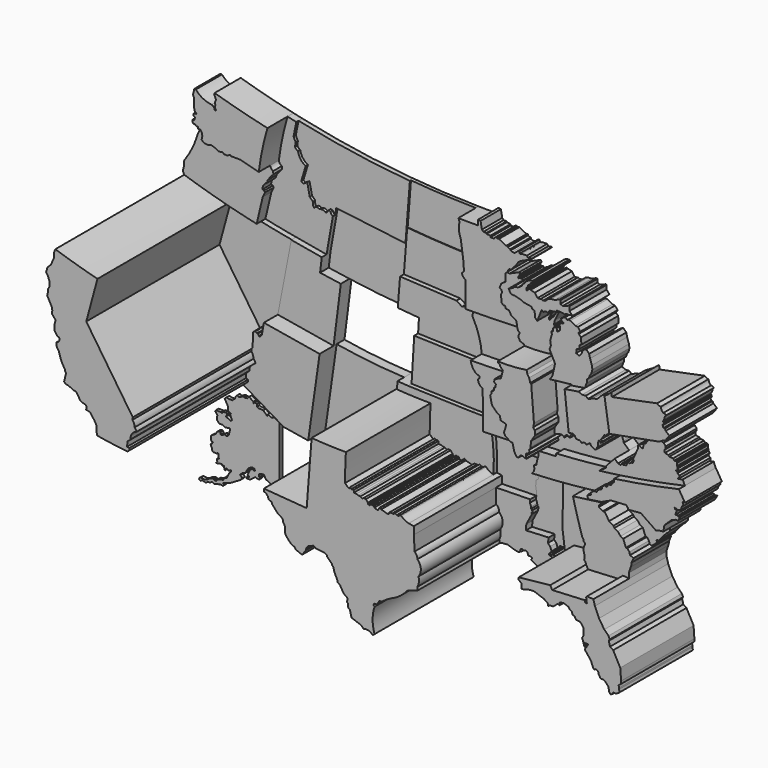
from build123d import *

# Parameters (mm, degrees)
F1_DEPTH  = 30.7990260072
F2_DEPTH  = 3.1576888498
F3_DEPTH  = 5.6013147348
F4_DEPTH  = 2.2417902341
F5_DEPTH  = 1.2953027168
F6_DEPTH  = 0.8156544997
F7_DEPTH  = 5.324292783
F8_DEPTH  = 0.4681481527
F9_DEPTH  = 1.5012963243
F10_DEPTH = 0.5812244861
F11_DEPTH = 0.6788332209
F12_DEPTH = 2.3252072804
F13_DEPTH = 1.6754652934
F14_DEPTH = 3.0938154048
F15_DEPTH = 21.2503264278
F16_DEPTH = 4.3551120624
F17_DEPTH = 2.4830561694
F18_DEPTH = 4.8563093416
F19_DEPTH = 2.377767066
F20_DEPTH = 3.7164258209
F21_DEPTH = 4.6140969189
F22_DEPTH = 10.3504074489
F23_DEPTH = 7.9508342104
F24_DEPTH = 5.2795218345
F25_DEPTH = 3.5314871415
F26_DEPTH = 5.2193226572
F27_DEPTH = 2.4033447262
F28_DEPTH = 9.296795703
F29_DEPTH = 3.8837500302
F30_DEPTH = 15.7101340571
F31_DEPTH = 0.590656419
F32_DEPTH = 1.1281150974
F33_DEPTH = 8.0284052098
F34_DEPTH = 3.8364393133
F35_DEPTH = 7.912619576
F36_DEPTH = 6.6369866053
F37_DEPTH = 1.4903000355
F38_DEPTH = 10.2310009529
F39_DEPTH = 2.3307632747


# Not quite as in the source:
# - a length typed as a fraction of an inch, garbled in the dataset ("3 / 203.2 mm" for 3/8 in), is restored


with BuildPart() as f1:
    # F0 (on Front) → F1 (new body)
    with BuildSketch(Plane.XZ):
        with BuildLine():
            ThreePointArc((-55.76618642, -11.2746760812), (-53.2719413055, -11.656261202), (-50.7680511674, -11.9683510489))
            ThreePointArc((-50.7680511674, -11.9683510489), (-50.3193289345, -11.8369929719), (-50.2125895868, -11.3817860976))
            Line((-50.2125895868, -11.3817860976), (-50.5702267274, -11.2950869668))
            Line((-50.5702267274, -11.2950869668), (-50.5268777232, -10.4118358553))
            ThreePointArc((-50.5268777232, -10.4118358553), (-50.2371740366, -10.2458641222), (-50.00888024, -10.0022316438))
            ThreePointArc((-50.00888024, -10.0022316438), (-49.7416635009, -9.0828643223), (-48.9668926341, -8.520395513))
            ThreePointArc((-48.9668926341, -8.520395513), (-49.0788735426, -8.20912138), (-49.285844705, -7.9510627672))
            ThreePointArc((-49.285844705, -7.9510627672), (-49.3812502891, -7.4127934878), (-49.6463008551, -6.9346886456))
            Line((-49.6463008551, -6.9346886456), (-49.6020540771, -6.5375023281))
            Line((-49.6020540771, -6.5375023281), (-57.5777995283, 5.3293358414))
            Line((-57.5777995283, 5.3293358414), (-55.6576036439, 12.389255143))
            ThreePointArc((-55.6576036437, 12.3892551435), (-59.2901733749, 13.3986211145), (-62.8919645981, 14.5128394504))
            Line((-62.8919645983, 14.51283945), (-63.0735483116, 14.0291548785))
            Line((-63.0735483116, 14.0291548785), (-63.0735483116, 13.1907441978))
            Line((-63.0735483116, 13.1907441978), (-63.6567825224, 11.9149022479))
            Line((-63.6567825224, 11.9149022479), (-63.9894166648, 11.618724452))
            Line((-63.9894166648, 11.618724452), (-64.025866278, 11.4592439277))
            Line((-64.025866278, 11.4592439277), (-64.2172447027, 11.4000088174))
            Line((-64.2172447027, 11.4000088174), (-64.4678537488, 10.5297024807))
            Line((-64.4678537488, 10.5297024807), (-64.162565794, 10.1150544642))
            Line((-64.162565794, 10.1150544642), (-63.8783530774, 9.2891879269))
            Line((-63.8783530774, 9.2891879269), (-63.9088953395, 8.4906866548))
            Line((-63.9088953395, 8.4906866548), (-64.1096106109, 8.1677956018))
            Line((-64.1096106109, 8.1677956018), (-64.1619687745, 7.5220134956))
            Line((-64.1619687745, 7.5220134956), (-64.2810001037, 7.0987103793))
            Line((-64.2810001037, 7.0987103793), (-63.5685403431, 5.7347760661))
            ThreePointArc((-63.5685403431, 5.7347760661), (-63.4185930064, 5.2825859598), (-63.4448181462, 4.8069050394))
            Line((-63.4448181462, 4.8069050394), (-63.4448181462, 4.5451978267))
            Line((-63.4448181462, 4.5451978267), (-62.8411102057, 3.8499890688))
            Line((-62.8411102057, 3.8499890688), (-63.0149865316, 3.1443933494))
            Line((-63.0149865316, 3.1443933494), (-63.0149865316, 2.1728543282))
            Line((-63.0149865316, 2.1728543282), (-62.5324151996, 1.4930982199))
            Line((-62.5324151996, 1.4930982199), (-62.2625893069, 1.4308303178))
            ThreePointArc((-62.2625893069, 1.4308303178), (-62.231252411, 0.900537109), (-62.6384180451, 0.5593494266))
            Line((-62.6384180451, 0.5593494266), (-62.6984674276, 0.0609399773))
            Line((-62.6984674276, 0.0609399773), (-62.5976392528, -0.2316117574))
            Line((-62.5976392528, -0.2316117574), (-62.2874800834, -0.6968475106))
            Line((-62.2874800834, -0.6968475106), (-61.8318060522, -2.0886206911))
            Line((-61.8318060522, -2.0886206911), (-61.2512876069, -3.078350151))
            Line((-61.2512876069, -3.078350151), (-61.2512876069, -3.344815845))
            Line((-61.2512876069, -3.344815845), (-61.0799878916, -3.4970816352))
            Line((-61.0799878916, -3.4970816352), (-61.0799878916, -3.7397557644))
            Line((-61.0799878916, -3.7397557644), (-61.3797635157, -4.9769176945))
            Line((-61.3797635157, -4.9769176945), (-61.0813804236, -5.2725109164))
            Line((-61.0813804236, -5.2725109164), (-60.6517408476, -5.3242747649))
            Line((-60.6517408476, -5.3242747649), (-59.7857258693, -5.743006249))
            Line((-59.7857258693, -5.743006249), (-59.3907862305, -5.7905893786))
            Line((-59.3907862305, -5.7905893786), (-59.0529450005, -6.1807713778))
            Line((-59.0529450005, -6.1807713778), (-58.634214358, -6.9325850496))
            Line((-58.634214358, -6.9325850496), (-58.225372693, -7.1437201073))
            Line((-58.225372693, -7.1437201073), (-57.6925463723, -7.2423345258))
            Line((-57.6925463723, -7.2423345258), (-57.5396531228, -7.4716729208))
            Line((-57.5396531228, -7.4716729208), (-57.4980767178, -7.7996421733))
            Line((-57.4980767178, -7.7996421733), (-57.5986637897, -7.8667006537))
            Line((-57.5986637897, -7.8667006537), (-57.5986637897, -7.9988630458))
            Line((-57.5986637897, -7.9988630458), (-56.9413812022, -8.1148542887))
            Line((-56.9413812022, -8.1148542887), (-56.4774117417, -8.8108039905))
            Line((-56.4774117417, -8.8108039905), (-56.2454315004, -9.0298989345))
            Line((-56.2454315004, -9.0298989345), (-55.8201291542, -9.8160636733))
            Line((-55.8201291542, -9.8160636733), (-55.76618642, -11.2746760812))
        make_face()
    extrude(amount=F1_DEPTH)

    # F0 (on Front) → F2 (join)
    with BuildSketch(Plane.XZ):
        with BuildLine():
            ThreePointArc((-55.6576036437, 12.3892551435), (-53.0704788693, 11.7388914273), (-50.470561214, 11.141718297))
            Line((-50.4705612141, 11.1417182965), (-49.4456978054, 15.5158490874))
            Line((-49.4456978054, 15.5158490874), (-49.0553502791, 16.3386766607))
            Line((-49.0553502791, 16.3386766607), (-49.1783767014, 16.596123376))
            Line((-49.1783767014, 16.596123376), (-49.4882253467, 16.6713063143))
            ThreePointArc((-49.4882253467, 16.6713063143), (-49.2826347673, 17.3879822948), (-48.7339921747, 17.8928419316))
            ThreePointArc((-48.7339921747, 17.8928419316), (-48.6278241804, 18.1031289), (-48.6024817907, 18.3373297014))
            ThreePointArc((-48.6024817912, 18.3373297017), (-48.1281044265, 18.9689623998), (-47.6061998447, 19.5619289729))
            Line((-47.6061998443, 19.5619289725), (-47.6660095299, 20.0164740546))
            ThreePointArc((-47.6660095299, 20.0164740546), (-47.996468492, 20.3020168152), (-48.167815662, 20.7037355491))
            Line((-48.167815662, 20.7037355491), (-51.3554645149, 21.54792116))
            Line((-51.3554645149, 21.54792116), (-53.0449175527, 21.54792116))
            Line((-53.0449175527, 21.54792116), (-53.0449175527, 21.6747900538))
            Line((-53.0449175527, 21.6747900538), (-53.6088720727, 21.4569475041))
            Line((-53.6088720727, 21.4569475041), (-54.0937461943, 21.4569475041))
            Line((-54.0937461943, 21.4569475041), (-54.431053249, 21.6958720252))
            Line((-54.431053249, 21.6958720252), (-54.5715952365, 21.6115463838))
            Line((-54.5715952365, 21.6115463838), (-55.0705284947, 21.6115463838))
            ThreePointArc((-55.0705284947, 21.6115463838), (-55.7229825425, 21.9411248455), (-56.4267773037, 22.1385866928))
            ThreePointArc((-56.4267773037, 22.1385866928), (-57.261991473, 21.9879443618), (-57.9797911798, 22.4407571283))
            ThreePointArc((-57.9797911798, 22.4407571283), (-57.858664179, 23.1740643492), (-58.1678747749, 23.8499341872))
            Line((-58.1678747749, 23.8499341872), (-58.5826193021, 23.8499341872))
            Line((-58.5826193021, 23.8499341872), (-58.5826193021, 24.1537071488))
            Line((-58.5826193021, 24.1537071488), (-58.8339331006, 24.1537071488))
            Line((-58.8339331006, 24.1537071488), (-59.5373567686, 23.9973261883))
            ThreePointArc((-59.5373567686, 23.9973261883), (-59.991386603, 22.6959778958), (-60.5588571781, 21.4399414254))
            ThreePointArc((-60.5588571781, 21.4399414254), (-61.5315761403, 18.9463261018), (-62.9081469696, 16.6508191179))
            Line((-62.9081469696, 16.6508191179), (-62.9741198717, 15.6869782258))
            Line((-62.9741198717, 15.6869782258), (-63.1382239307, 15.013601922))
            Line((-63.1382239307, 15.013601922), (-62.8919645983, 14.51283945))
            ThreePointArc((-62.8919645981, 14.5128394504), (-59.2901733749, 13.3986211145), (-55.6576036437, 12.3892551435))
        make_face()
    extrude(amount=F2_DEPTH)

    # F0 (on Front) → F3 (join)
    with BuildSketch(Plane.XZ):
        with BuildLine():
            ThreePointArc((-48.167815662, 20.7037355491), (-47.5651659137, 24.291276367), (-46.6767078818, 27.8189212137))
            ThreePointArc((-46.6767078818, 27.8189212137), (-51.197937914, 28.9224786313), (-55.683079851, 30.1645985063))
            Line((-55.683079851, 30.1645985063), (-55.7523696824, 30.1669012844))
            Line((-55.7523696824, 30.1669012844), (-55.8090910263, 29.9923650948))
            Line((-55.8090910263, 29.9923650948), (-55.4694318045, 29.181819066))
            ThreePointArc((-55.4694318045, 29.181819066), (-55.6422043168, 28.8069079271), (-55.5835882223, 28.3982848041))
            ThreePointArc((-55.5835882223, 28.3982848041), (-55.6690874012, 28.0652968341), (-55.5109448615, 27.7600395084))
            Line((-55.5109448615, 27.7600395084), (-55.5109448615, 27.5680483532))
            Line((-55.5109448615, 27.5680483532), (-55.7054969163, 27.5751250545))
            ThreePointArc((-55.7054969163, 27.5751250545), (-55.8744616782, 27.9979531139), (-56.2517697828, 28.2528477053))
            ThreePointArc((-56.2517697828, 28.2528477053), (-57.7362703024, 28.6947121918), (-58.9524616764, 29.6538078902))
            Line((-58.9524616764, 29.6538078902), (-59.2099027806, 29.6799892165))
            Line((-59.2099027806, 29.6799892165), (-59.4149812323, 28.8073082683))
            Line((-59.4149812323, 28.8073082683), (-59.4149812323, 28.624045718))
            Line((-59.4149812323, 28.624045718), (-59.2284494923, 28.3055178453))
            Line((-59.2284494923, 28.3055178453), (-59.2284494923, 27.3559227732))
            Line((-59.2284494923, 27.3559227732), (-59.2981808709, 27.1056971299))
            Line((-59.2981808709, 27.1056971299), (-59.1569251532, 26.3356362072))
            Line((-59.1569251532, 26.3356362072), (-58.8031259952, 25.9909494525))
            Line((-58.8031259952, 25.9909494525), (-59.3043485763, 25.9408267455))
            Line((-59.3043485763, 25.9408267455), (-59.3426251591, 25.5483829177))
            Line((-59.3426251591, 25.5483829177), (-59.0705368766, 25.4003355417))
            Line((-59.0705368766, 25.4003355417), (-59.2488122938, 24.9278978306))
            Line((-59.2488122938, 24.9278978306), (-59.5342055828, 24.9278978306))
            Line((-59.5342055828, 24.9278978306), (-59.5722487444, 24.5992430703))
            Line((-59.5722487444, 24.5992430703), (-59.3147509395, 24.3054086978))
            Line((-59.3147509395, 24.3054086978), (-59.1333361486, 24.3824935601))
            Line((-59.1333361486, 24.3824935601), (-58.8339331006, 24.1537071488))
            Line((-58.8339331006, 24.1537071488), (-58.5826193021, 24.1537071488))
            Line((-58.5826193021, 24.1537071488), (-58.5826193021, 23.8499341872))
            Line((-58.5826193021, 23.8499341872), (-58.1678747749, 23.8499341872))
            ThreePointArc((-58.1678747749, 23.8499341872), (-57.858664179, 23.1740643492), (-57.9797911798, 22.4407571283))
            ThreePointArc((-57.9797911798, 22.4407571283), (-57.261991473, 21.9879443618), (-56.4267773037, 22.1385866928))
            ThreePointArc((-56.4267773037, 22.1385866928), (-55.7229825425, 21.9411248455), (-55.0705284947, 21.6115463838))
            Line((-55.0705284947, 21.6115463838), (-54.5715952365, 21.6115463838))
            Line((-54.5715952365, 21.6115463838), (-54.431053249, 21.6958720252))
            Line((-54.431053249, 21.6958720252), (-54.0937461943, 21.4569475041))
            Line((-54.0937461943, 21.4569475041), (-53.6088720727, 21.4569475041))
            Line((-53.6088720727, 21.4569475041), (-53.0449175527, 21.6747900538))
            Line((-53.0449175527, 21.6747900538), (-53.0449175527, 21.54792116))
            Line((-53.0449175527, 21.54792116), (-51.3554645149, 21.54792116))
            Line((-51.3554645149, 21.54792116), (-48.167815662, 20.7037355491))
        make_face()
    extrude(amount=F3_DEPTH)

    # F0 (on Front) → F4 (join)
    with BuildSketch(Plane.XZ):
        with BuildLine():
            Line((-47.8545420126, -3.9132098561), (-47.508448233, -1.9300360594))
            Line((-47.508448233, -1.9300360594), (-45.2000181328, 10.1014599256))
            ThreePointArc((-45.2000181327, 10.1014599261), (-47.8406606081, 10.5943768883), (-50.470561214, 11.141718297))
            ThreePointArc((-50.470561214, 11.141718297), (-53.0704788693, 11.7388914273), (-55.6576036437, 12.3892551435))
            Line((-55.6576036439, 12.389255143), (-57.5777995283, 5.3293358414))
            Line((-57.5777995283, 5.3293358414), (-49.6020540771, -6.5375023281))
            Line((-49.6020540771, -6.5375023281), (-49.447282376, -6.308706939))
            Line((-49.447282376, -6.308706939), (-49.342866803, -3.9132098561))
            ThreePointArc((-49.342866803, -3.9132098561), (-49.1740222372, -3.8075852222), (-48.9796634653, -3.7641143294))
            ThreePointArc((-48.9796634653, -3.7641143294), (-48.8371354256, -3.8218019803), (-48.7134960006, -3.9132098561))
            ThreePointArc((-48.7134960006, -3.9132098561), (-48.6196831353, -3.9124596116), (-48.5258702701, -3.9132098561))
            ThreePointArc((-48.5258702701, -3.9132098561), (-48.4322724661, -4.0609582684), (-48.3734417584, -4.2256673758))
            ThreePointArc((-48.3734417584, -4.2256673758), (-48.2529665845, -4.2564015361), (-48.1295615263, -4.241234211))
            ThreePointArc((-48.1295615263, -4.241234211), (-48.0154508631, -4.0576039556), (-47.8545420126, -3.9132098561))
        make_face()
    extrude(amount=F4_DEPTH)

    # F0 (on Front) → F5 (join)
    with BuildSketch(Plane.XZ):
        with BuildLine():
            ThreePointArc((-50.470561214, 11.141718297), (-47.8406606081, 10.5943768883), (-45.2000181327, 10.1014599261))
            Line((-45.2000181328, 10.1014599256), (-39.9818273184, 9.1830576061))
            Line((-39.9818273184, 9.1830576061), (-38.9115960638, 15.2639121327))
            ThreePointArc((-38.9115960638, 15.2639121327), (-39.1717820192, 15.5335304075), (-39.3172346083, 15.8788335928))
            ThreePointArc((-39.3172346083, 15.8788335928), (-39.5256135255, 15.943257871), (-39.7377114207, 15.8923978315))
            ThreePointArc((-39.7377114207, 15.8923978315), (-39.8585232316, 15.6062940352), (-40.144627361, 15.4854830134))
            ThreePointArc((-40.144627361, 15.4854830134), (-40.6775045734, 15.7063659375), (-41.2432959109, 15.5939935568))
            ThreePointArc((-41.2432959109, 15.5939935568), (-41.705714351, 15.7667568095), (-42.1113780132, 15.4854830134))
            ThreePointArc((-42.1113780132, 15.4854830134), (-42.3069241226, 15.9217981908), (-42.3308702221, 16.3993291313))
            Line((-42.3308702221, 16.3993291313), (-42.8677366645, 16.9361955737))
            Line((-42.8677366645, 16.9361955737), (-43.2853002011, 18.9941858472))
            Line((-43.2853002011, 18.9941858472), (-44.0011221243, 18.546796023))
            Line((-44.0011221243, 18.546796023), (-44.3292090428, 18.830142388))
            Line((-44.3292090428, 18.830142388), (-43.5583446126, 21.3654890505))
            ThreePointArc((-43.5583446126, 21.3654890505), (-44.4498033761, 22.1140503933), (-44.8796206462, 23.1958544074))
            ThreePointArc((-44.8796206462, 23.1958544074), (-45.1848735264, 23.3819773402), (-45.3948844084, 23.6713153716))
            Line((-45.3948844084, 23.6713153716), (-45.2845300623, 24.3886163769))
            Line((-45.2845300623, 24.3886163769), (-45.6431816872, 25.1335059689))
            Line((-45.6431816872, 25.1335059689), (-45.1704363674, 27.4838002688))
            ThreePointArc((-45.1704363674, 27.4838002688), (-45.9239994515, 27.6494400309), (-46.6767078818, 27.8189212137))
            ThreePointArc((-46.6767078818, 27.8189212137), (-47.5651659137, 24.291276367), (-48.167815662, 20.7037355491))
            ThreePointArc((-48.167815662, 20.7037355491), (-47.996468492, 20.3020168152), (-47.6660095299, 20.0164740546))
            Line((-47.6660095299, 20.0164740546), (-47.6061998443, 19.5619289725))
            ThreePointArc((-47.6061998447, 19.5619289729), (-48.1281044265, 18.9689623998), (-48.6024817912, 18.3373297017))
            ThreePointArc((-48.6024817907, 18.3373297014), (-48.6278241804, 18.1031289), (-48.7339921747, 17.8928419316))
            ThreePointArc((-48.7339921747, 17.8928419316), (-49.2826347673, 17.3879822948), (-49.4882253467, 16.6713063143))
            Line((-49.4882253467, 16.6713063143), (-49.1783767014, 16.596123376))
            Line((-49.1783767014, 16.596123376), (-49.0553502791, 16.3386766607))
            Line((-49.0553502791, 16.3386766607), (-49.4456978054, 15.5158490874))
            Line((-49.4456978054, 15.5158490874), (-50.4705612141, 11.1417182965))
        make_face()
    extrude(amount=F5_DEPTH)

    # F0 (on Front) → F6 (join)
    with BuildSketch(Plane.XZ):
        with BuildLine():
            Line((-38.7098662514, 16.4101033301), (-26.8373622723, 14.9476111457))
            Line((-26.8373622723, 14.9476111457), (-26.6511585405, 17.3206204985))
            Line((-26.6511585405, 17.3206204985), (-26.080011565, 24.5994064863))
            ThreePointArc((-26.0800115651, 24.5994064856), (-35.6712894804, 25.7367177408), (-45.1704363674, 27.4838002688))
            Line((-45.1704363674, 27.4838002688), (-45.6431816872, 25.1335059689))
            Line((-45.6431816872, 25.1335059689), (-45.2845300623, 24.3886163769))
            Line((-45.2845300623, 24.3886163769), (-45.3948844084, 23.6713153716))
            ThreePointArc((-45.3948844084, 23.6713153716), (-45.1848735264, 23.3819773402), (-44.8796206462, 23.1958544074))
            ThreePointArc((-44.8796206462, 23.1958544074), (-44.4498033761, 22.1140503933), (-43.5583446126, 21.3654890505))
            Line((-43.5583446126, 21.3654890505), (-44.3292090428, 18.830142388))
            Line((-44.3292090428, 18.830142388), (-44.0011221243, 18.546796023))
            Line((-44.0011221243, 18.546796023), (-43.2853002011, 18.9941858472))
            Line((-43.2853002011, 18.9941858472), (-42.8677366645, 16.9361955737))
            Line((-42.8677366645, 16.9361955737), (-42.3308702221, 16.3993291313))
            ThreePointArc((-42.3308702221, 16.3993291313), (-42.3069241226, 15.9217981908), (-42.1113780132, 15.4854830134))
            ThreePointArc((-42.1113780132, 15.4854830134), (-41.705714351, 15.7667568095), (-41.2432959109, 15.5939935568))
            ThreePointArc((-41.2432959109, 15.5939935568), (-40.6775045734, 15.7063659375), (-40.144627361, 15.4854830134))
            ThreePointArc((-40.144627361, 15.4854830134), (-39.8585232316, 15.6062940352), (-39.7377114207, 15.8923978315))
            ThreePointArc((-39.7377114207, 15.8923978315), (-39.5256135255, 15.943257871), (-39.3172346083, 15.8788335928))
            ThreePointArc((-39.3172346083, 15.8788335928), (-39.1717820192, 15.5335304075), (-38.9115960638, 15.2639121327))
            Line((-38.9115960638, 15.2639121327), (-38.7098662514, 16.4101033301))
        make_face()
    extrude(amount=F6_DEPTH)

    # F0 (on Front) → F8 (join)
    with BuildSketch(Plane.XZ):
        Polygon((-31.6450474466, 5.5908797214), (-27.6139397174, 5.2254982293), (-27.2187964607, 10.0865544546), (-26.8373622723, 14.9476111457), (-38.7098662514, 16.4101033301), (-38.9115960638, 15.2639121327), (-39.9818273184, 9.1830576061), (-40.2666280768, 6.7584350603), (-36.7156277562, 6.231837466), align=None)
    extrude(amount=F8_DEPTH)

    # F0 (on Front) → F9 (join)
    with BuildSketch(Plane.XZ):
        with BuildLine():
            Line((-23.9753960315, 4.920837575), (-24.1286147911, 2.4957993984))
            Line((-24.1286147911, 2.4957993984), (-11.71705725, 2.1274687859))
            ThreePointArc((-11.71705725, 2.1274687859), (-12.1884943161, 2.8127988837), (-12.4263753705, 3.609882853))
            ThreePointArc((-12.426375371, 3.609882853), (-12.8579294834, 5.9923830438), (-13.7437965887, 8.2457772798))
            ThreePointArc((-13.7437965882, 8.24577728), (-14.1105528443, 8.3512707161), (-14.3010127554, 8.6819730577))
            ThreePointArc((-14.3010127554, 8.6819730577), (-15.4045802774, 9.1582246432), (-16.5932967209, 8.9803762102))
            Line((-16.5932967209, 8.9803762102), (-17.528714097, 9.599598803))
            Line((-17.528714097, 9.599598803), (-27.2187964607, 10.0865544546))
            Line((-27.2187964607, 10.0865544546), (-27.6139397174, 5.2254982293))
            Line((-27.6139397174, 5.2254982293), (-23.9753960315, 4.920837575))
        make_face()
    extrude(amount=F9_DEPTH)

    # F0 (on Front) → F10 (join)
    with BuildSketch(Plane.XZ):
        with BuildLine():
            Line((-26.080011565, 24.5994064863), (-26.6511585405, 17.3206204985))
            ThreePointArc((-26.6511585405, 17.3206204985), (-20.3320219172, 16.8697697188), (-14.0008219109, 16.64469069))
            Line((-14.0008219109, 16.64469069), (-14.0692586408, 17.7708378492))
            Line((-14.0692586408, 17.7708378492), (-14.5167611901, 21.0284715279))
            ThreePointArc((-14.5167611901, 21.0284715279), (-14.8158392328, 22.1196391511), (-14.7923138146, 23.2508071371))
            ThreePointArc((-14.7923138146, 23.2508071371), (-14.779164463, 23.6714548147), (-14.9612011933, 24.0509017846))
            ThreePointArc((-14.9612011933, 24.0509017846), (-20.5256538645, 24.2228359013), (-26.0800115651, 24.5994064856))
        make_face()
    extrude(amount=F10_DEPTH)

    # F0 (on Front) → F11 (join)
    with BuildSketch(Plane.XZ):
        with BuildLine():
            ThreePointArc((-14.3010127554, 8.6819730577), (-14.1105528443, 8.3512707161), (-13.7437965882, 8.24577728))
            Line((-13.7437965882, 8.24577728), (-14.046258424, 8.8379064071))
            Line((-14.046258424, 8.8379064071), (-13.7437965882, 9.9637021588))
            ThreePointArc((-13.7437965882, 9.9637021588), (-13.9655317102, 10.3199110397), (-13.9587224955, 10.7394403781))
            ThreePointArc((-13.9587224955, 10.7394403781), (-13.8516885082, 10.7392743739), (-13.7446544463, 10.7391668523))
            ThreePointArc((-13.7446544463, 10.7391668523), (-13.6772495598, 12.9465201983), (-13.7200684287, 15.1544873081))
            ThreePointArc((-13.7200684287, 15.1544873081), (-14.1309257699, 15.4983575763), (-14.338689513, 15.9922044586))
            ThreePointArc((-14.338689513, 15.9922044586), (-14.0404762204, 16.2515046264), (-14.0008219109, 16.64469069))
            ThreePointArc((-14.0008219109, 16.64469069), (-20.3320219172, 16.8697697188), (-26.6511585405, 17.3206204985))
            Line((-26.6511585405, 17.3206204985), (-26.8373622723, 14.9476111457))
            Line((-26.8373622723, 14.9476111457), (-27.2187964607, 10.0865544546))
            Line((-27.2187964607, 10.0865544546), (-17.528714097, 9.599598803))
            Line((-17.528714097, 9.599598803), (-16.5932967209, 8.9803762102))
            ThreePointArc((-16.5932967209, 8.9803762102), (-15.4045802774, 9.1582246432), (-14.3010127554, 8.6819730577))
        make_face()
    extrude(amount=F11_DEPTH)

    # F0 (on Front) → F12 (join)
    with BuildSketch(Plane.XZ):
        with BuildLine():
            Line((-13.6910863221, -5.2475701086), (-10.3551703365, -5.2687089489))
            ThreePointArc((-10.3551703365, -5.2687089489), (-10.2955350096, -2.610484202), (-10.4355542734, 0.0447200807))
            ThreePointArc((-10.4355542734, 0.0447200807), (-10.9657571067, 0.5220318102), (-11.1632015665, 1.2075660666))
            ThreePointArc((-11.1632015665, 1.2075660666), (-10.9201031487, 1.4316607477), (-10.9997018215, 1.7525646556))
            ThreePointArc((-10.9997018215, 1.7525646556), (-11.3901872705, 1.8791546246), (-11.71705725, 2.1274687859))
            Line((-11.71705725, 2.1274687859), (-24.1286147911, 2.4957993984))
            Line((-24.1286147911, 2.4957993984), (-24.5903491224, -4.9049796536))
            Line((-24.5903491224, -4.9049796536), (-13.6910863221, -5.2475701086))
        make_face()
    extrude(amount=F12_DEPTH)



with BuildPart() as f7:
    # F0 (on Front) → F7 (new body)
    with BuildSketch(Plane.XZ):
        with BuildLine():
            Line((-39.9094208906, -17.2505455833), (-37.950155588, -3.534442087))
            Line((-37.950155588, -3.534442087), (-47.508448233, -1.9300360593))
            Line((-47.508448233, -1.9300360594), (-47.8545420126, -3.9132098561))
            ThreePointArc((-47.8545420126, -3.9132098561), (-48.0154508631, -4.0576039556), (-48.1295615263, -4.241234211))
            ThreePointArc((-48.1295615263, -4.241234211), (-48.2529665845, -4.2564015361), (-48.3734417584, -4.2256673758))
            ThreePointArc((-48.3734417584, -4.2256673758), (-48.4322724661, -4.0609582684), (-48.5258702701, -3.9132098561))
            ThreePointArc((-48.5258702701, -3.9132098561), (-48.6196831353, -3.9124596116), (-48.7134960006, -3.9132098561))
            ThreePointArc((-48.7134960006, -3.9132098561), (-48.8371354256, -3.8218019803), (-48.9796634653, -3.7641143294))
            ThreePointArc((-48.9796634653, -3.7641143294), (-49.1740222372, -3.8075852222), (-49.342866803, -3.9132098561))
            Line((-49.342866803, -3.9132098561), (-49.447282376, -6.308706939))
            Line((-49.447282376, -6.308706939), (-49.6020540771, -6.5375023281))
            Line((-49.6020540771, -6.5375023281), (-49.6463008551, -6.9346886456))
            ThreePointArc((-49.6463008551, -6.9346886456), (-49.3812502891, -7.4127934878), (-49.285844705, -7.9510627672))
            ThreePointArc((-49.285844705, -7.9510627672), (-49.0788735426, -8.20912138), (-48.9668926341, -8.520395513))
            ThreePointArc((-48.9668926341, -8.520395513), (-49.7416635009, -9.0828643223), (-50.00888024, -10.0022316438))
            ThreePointArc((-50.00888024, -10.0022316438), (-50.2371740366, -10.2458641222), (-50.5268777232, -10.4118358553))
            Line((-50.5268777232, -10.4118358553), (-50.5702267274, -11.2950869668))
            Line((-50.5702267274, -11.2950869668), (-50.2125895868, -11.3817860976))
            ThreePointArc((-50.2125895868, -11.3817860976), (-50.3193289345, -11.8369929719), (-50.7680511674, -11.9683510489))
            ThreePointArc((-50.7680511674, -11.9683510489), (-50.9148498137, -12.2104011444), (-51.0436093454, -12.4625103952))
            Line((-51.0436093454, -12.4625103952), (-44.1081681743, -16.5658906881))
            Line((-44.1081681743, -16.5658906881), (-39.9094208906, -17.2505455833))
        make_face()
    extrude(amount=F7_DEPTH)

    # F0 (on Front) → F13 (join)
    with BuildSketch(Plane.XZ):
        with BuildLine():
            Line((-26.4697589295, -6.0503290105), (-26.3802006479, -4.7795181348))
            ThreePointArc((-26.3802006479, -4.7795181348), (-32.1835807884, -4.3279881939), (-37.950155588, -3.5344420871))
            Line((-37.950155588, -3.534442087), (-39.9094208906, -17.2505455833))
            Line((-39.9094208906, -17.2505455833), (-38.2098778531, -17.4933153834))
            Line((-38.2098778531, -17.4933153834), (-38.0887524668, -16.351234113))
            Line((-38.0887524668, -16.351234113), (-34.7779492615, -16.8088237689))
            Line((-34.7779492615, -16.8088237689), (-34.7779492615, -16.351234113))
            Line((-34.7779492615, -16.351234113), (-27.4295837995, -16.9164926494))
            Line((-27.4295837995, -16.9164926494), (-26.5850581333, -6.0413752555))
            Line((-26.5850581333, -6.0413752555), (-26.4697589295, -6.0503290105))
        make_face()
    extrude(amount=F13_DEPTH)


with BuildPart() as f1_1:
    add(f1.part)

    add(f7.part)  # F14 merges F7
    # F0 (on Front) → F14 (join)
    with BuildSketch(Plane.XZ):
        with BuildLine():
            ThreePointArc((-11.1884486494, -12.8134557549), (-10.6148592297, -13.273076286), (-9.9221188926, -13.5187726033))
            ThreePointArc((-9.9221188926, -13.5187726033), (-9.9190205581, -9.9784053679), (-10.3551703365, -6.4650048596))
            Line((-10.3551703365, -6.4650048596), (-10.3551703365, -5.2687089489))
            Line((-10.3551703365, -5.2687089489), (-13.6910863221, -5.2475701086))
            Line((-13.6910863221, -5.2475701086), (-24.5903491224, -4.9049796536))
            Line((-24.5903491224, -4.9049796536), (-26.3802006479, -4.7795181348))
            Line((-26.3802006479, -4.7795181348), (-26.4697589295, -6.0503290105))
            ThreePointArc((-26.4697589295, -6.0503290105), (-23.5919359097, -6.2180075309), (-20.7097856248, -6.274497834))
            ThreePointArc((-20.7097856248, -6.274497834), (-20.8127796793, -8.6395362508), (-20.8651330308, -11.006237249))
            Line((-20.8651330308, -11.006237249), (-20.2424753315, -11.5705867895))
            Line((-20.2424753315, -11.5705867895), (-20.1036335029, -11.5551607924))
            Line((-20.1036335029, -11.5551607924), (-20.0110719098, -11.3422683427))
            Line((-20.0110719098, -11.3422683427), (-19.8166926764, -11.5705867895))
            Line((-19.8166926764, -11.5705867895), (-19.6377405623, -11.5551607924))
            Line((-19.6377405623, -11.5551607924), (-19.6068863238, -11.4224889138))
            Line((-19.6068863238, -11.4224889138), (-19.3631407578, -11.5335626011))
            Line((-19.3631407578, -11.5335626011), (-19.3505607035, -11.9647318985))
            Line((-19.3505607035, -11.9647318985), (-18.8941908977, -11.9949812619))
            Line((-18.8941908977, -11.9949812619), (-18.6248182344, -12.1244079797))
            Line((-18.6248182344, -12.1244079797), (-18.2304611726, -12.1593019088))
            Line((-18.2304611726, -12.1593019088), (-17.8836837274, -12.3959292514))
            Line((-17.8836837274, -12.3959292514), (-17.6615363527, -12.2077210902))
            Line((-17.6615363527, -12.2077210902), (-17.288203883, -12.272514542))
            Line((-17.288203883, -12.272514542), (-16.9333857519, -12.6674429587))
            Line((-16.9333857519, -12.6674429587), (-16.8901904914, -12.9081035497))
            Line((-16.8901904914, -12.9081035497), (-16.6310178062, -12.9914090958))
            Line((-16.6310178062, -12.9914090958), (-16.3471619546, -12.7291514356))
            Line((-16.3471619546, -12.7291514356), (-16.2443646188, -12.8014570091))
            Line((-16.2443646188, -12.8014570091), (-15.889945997, -12.8143445509))
            Line((-15.889945997, -12.8143445509), (-15.8190622726, -13.0688813571))
            Line((-15.8190622726, -13.0688813571), (-15.3133530673, -13.2623448612))
            Line((-15.3133530673, -13.2623448612), (-15.1554750692, -13.2011267932))
            Line((-15.1554750692, -13.2011267932), (-14.9331582397, -12.7726025616))
            Line((-14.9331582397, -12.7726025616), (-14.7946132376, -12.7597150198))
            Line((-14.7946132376, -12.7597150198), (-14.6625114452, -12.959266552))
            Line((-14.6625114452, -12.959266552), (-13.5384095268, -13.2817805401))
            Line((-13.5384095268, -13.2817805401), (-13.2854079137, -13.1552797336))
            Line((-13.2854079137, -13.1552797336), (-13.2206150229, -12.9331312367))
            Line((-13.2206150229, -12.9331312367), (-12.7454654741, -12.9207890925))
            Line((-12.7454654741, -12.9207890925), (-12.5371954368, -13.0230589862))
            ThreePointArc((-12.5371954368, -13.0230589862), (-12.2934597589, -12.8209286867), (-12.0086328402, -12.959266552))
            Line((-12.0086328402, -12.959266552), (-11.5894274998, -12.9774924808))
            ThreePointArc((-11.5894274998, -12.9774924808), (-11.4319611314, -12.7903065966), (-11.1884486494, -12.8134557549))
        make_face()
    extrude(amount=F14_DEPTH)

    # F0 (on Front) → F15 (join)
    with BuildSketch(Plane.XZ):
        with BuildLine():
            Line((-20.5434954945, -28.8220484329), (-20.3423066474, -28.9508093848))
            Line((-20.3423066474, -28.9508093848), (-20.3423066474, -29.3880655881))
            ThreePointArc((-20.3423066474, -29.3880655881), (-20.2500965735, -29.6594552549), (-20.0116397517, -29.8184942222))
            ThreePointArc((-20.0116397517, -29.8184942222), (-19.8946017501, -30.3979763947), (-19.7136506973, -30.9607855974))
            Line((-19.7136506973, -30.9607855974), (-18.140930688, -31.5236538112))
            Line((-18.140930688, -31.5236538112), (-17.6773921589, -31.9540802009))
            Line((-17.6773921589, -31.9540802009), (-17.4787327893, -31.9375274979))
            Line((-17.4787327893, -31.9375274979), (-17.2469635248, -31.871307708))
            Line((-17.2469635248, -31.871307708), (-16.6344304685, -31.9706373928))
            Line((-16.6344304685, -31.9706373928), (-16.1046721496, -32.3845110795))
            Line((-16.1046721496, -32.3845110795), (-15.7901281477, -32.152741815))
            ThreePointArc((-15.7901281477, -32.152741815), (-16.127503064, -30.0794130773), (-15.7901281477, -28.0060843397))
            Line((-15.7901281477, -28.0060843397), (-15.9742121609, -27.803414166))
            Line((-15.9742121609, -27.803414166), (-15.8488605048, -27.5777789404))
            Line((-15.8488605048, -27.5777789404), (-15.4059494492, -27.5359965513))
            Line((-15.4059494492, -27.5359965513), (-14.9463257747, -26.8587654316))
            Line((-14.9463257747, -26.8587654316), (-14.5827627664, -26.8587654316))
            ThreePointArc((-14.5827627664, -26.8587654316), (-13.7761643746, -26.2921774571), (-12.9187773248, -25.805854164))
            ThreePointArc((-12.9187773248, -25.805854164), (-11.4287794213, -24.9615001418), (-10.1886421003, -23.780362177))
            Line((-10.1886421003, -23.780362177), (-8.3537306416, -23.1224331924))
            Line((-8.3537306416, -23.1224331924), (-8.4524630263, -22.6287721105))
            ThreePointArc((-8.4524630263, -22.6287721105), (-8.1966791861, -21.8332664048), (-8.2549982569, -20.9996876223))
            ThreePointArc((-8.2549982569, -20.9996876223), (-7.8585251969, -19.696029901), (-8.4524630263, -18.4696726136))
            ThreePointArc((-8.4524630263, -18.4696726136), (-8.5679824902, -17.9015238358), (-8.9607635703, -17.4750724277))
            Line((-8.9607635703, -17.4750724277), (-9.011047146, -14.933791419))
            Line((-9.011047146, -14.933791419), (-9.0743189015, -13.6673418102))
            Line((-9.0743189015, -13.6673418102), (-9.9221188926, -13.5187726033))
            ThreePointArc((-9.9221188926, -13.5187726033), (-10.6148592297, -13.273076286), (-11.1884486494, -12.8134557549))
            ThreePointArc((-11.1884486494, -12.8134557549), (-11.4319611314, -12.7903065966), (-11.5894274998, -12.9774924808))
            Line((-11.5894274998, -12.9774924808), (-12.0086328402, -12.959266552))
            ThreePointArc((-12.0086328402, -12.959266552), (-12.2934597589, -12.8209286867), (-12.5371954368, -13.0230589862))
            Line((-12.5371954368, -13.0230589862), (-12.7454654741, -12.9207890925))
            Line((-12.7454654741, -12.9207890925), (-13.2206150229, -12.9331312367))
            Line((-13.2206150229, -12.9331312367), (-13.2854079137, -13.1552797336))
            Line((-13.2854079137, -13.1552797336), (-13.5384095268, -13.2817805401))
            Line((-13.5384095268, -13.2817805401), (-14.6625114452, -12.959266552))
            Line((-14.6625114452, -12.959266552), (-14.7946132376, -12.7597150198))
            Line((-14.7946132376, -12.7597150198), (-14.9331582397, -12.7726025616))
            Line((-14.9331582397, -12.7726025616), (-15.1554750692, -13.2011267932))
            Line((-15.1554750692, -13.2011267932), (-15.3133530673, -13.2623448612))
            Line((-15.3133530673, -13.2623448612), (-15.8190622726, -13.0688813571))
            Line((-15.8190622726, -13.0688813571), (-15.889945997, -12.8143445509))
            Line((-15.889945997, -12.8143445509), (-16.2443646188, -12.8014570091))
            Line((-16.2443646188, -12.8014570091), (-16.3471619546, -12.7291514356))
            Line((-16.3471619546, -12.7291514356), (-16.6310178062, -12.9914090958))
            Line((-16.6310178062, -12.9914090958), (-16.8901904914, -12.9081035497))
            Line((-16.8901904914, -12.9081035497), (-16.9333857519, -12.6674429587))
            Line((-16.9333857519, -12.6674429587), (-17.288203883, -12.272514542))
            Line((-17.288203883, -12.272514542), (-17.6615363527, -12.2077210902))
            Line((-17.6615363527, -12.2077210902), (-17.8836837274, -12.3959292514))
            Line((-17.8836837274, -12.3959292514), (-18.2304611726, -12.1593019088))
            Line((-18.2304611726, -12.1593019088), (-18.6248182344, -12.1244079797))
            Line((-18.6248182344, -12.1244079797), (-18.8941908977, -11.9949812619))
            Line((-18.8941908977, -11.9949812619), (-19.3505607035, -11.9647318985))
            Line((-19.3505607035, -11.9647318985), (-19.3631407578, -11.5335626011))
            Line((-19.3631407578, -11.5335626011), (-19.6068863238, -11.4224889138))
            Line((-19.6068863238, -11.4224889138), (-19.6377405623, -11.5551607924))
            Line((-19.6377405623, -11.5551607924), (-19.8166926764, -11.5705867895))
            Line((-19.8166926764, -11.5705867895), (-20.0110719098, -11.3422683427))
            Line((-20.0110719098, -11.3422683427), (-20.1036335029, -11.5551607924))
            Line((-20.1036335029, -11.5551607924), (-20.2424753315, -11.5705867895))
            Line((-20.2424753315, -11.5705867895), (-20.8651330308, -11.006237249))
            ThreePointArc((-20.8651330308, -11.006237249), (-20.8127796793, -8.6395362508), (-20.7097856248, -6.274497834))
            ThreePointArc((-20.7097856248, -6.274497834), (-23.5919359097, -6.2180075309), (-26.4697589295, -6.0503290105))
            Line((-26.4697589295, -6.0503290105), (-26.5850581333, -6.0413752555))
            Line((-26.5850581333, -6.0413752555), (-27.4295837995, -16.9164926494))
            Line((-27.4295837995, -16.9164926494), (-34.7779492615, -16.351234113))
            Line((-34.7779492615, -16.351234113), (-34.7779492615, -16.8088237689))
            Line((-34.7779492615, -16.8088237689), (-34.4752715839, -16.8751445583))
            Line((-34.4752715839, -16.8751445583), (-34.1131074193, -17.2547603219))
            Line((-34.1131074193, -17.2547603219), (-33.929844869, -17.7216430581))
            Line((-33.929844869, -17.7216430581), (-33.4585989526, -17.9354501148))
            Line((-33.4585989526, -17.9354501148), (-33.3276968103, -18.2583400457))
            Line((-33.3276968103, -18.2583400457), (-32.3502972906, -19.3840955511))
            Line((-32.3502972906, -19.3840955511), (-31.8268009434, -19.6493652421))
            Line((-31.8268009434, -19.6493652421), (-31.5397355507, -19.9364295125))
            Line((-31.5397355507, -19.9364295125), (-31.4713880372, -20.3146256714))
            Line((-31.4713880372, -20.3146256714), (-31.1271003932, -20.9344484975))
            Line((-31.1271003932, -20.9344484975), (-31.1068919053, -21.9557650162))
            Line((-31.1068919053, -21.9557650162), (-30.8538162259, -22.3921054903))
            Line((-30.8538162259, -22.3921054903), (-30.0922886424, -23.202790674))
            Line((-30.0922886424, -23.202790674), (-29.5090454539, -23.4579581662))
            Line((-29.5090454539, -23.4579581662), (-29.262990365, -23.7951440213))
            Line((-29.262990365, -23.7951440213), (-28.2240911007, -24.2143504839))
            Line((-28.2240911007, -24.2143504839), (-27.5284713308, -23.2694391508))
            Line((-27.5284713308, -23.2694391508), (-27.4935636439, -22.9640030633))
            Line((-27.4935636439, -22.9640030633), (-27.1673665391, -22.5590532475))
            Line((-27.1673665391, -22.5590532475), (-26.2355806578, -22.1918929721))
            Line((-26.2355806578, -22.1918929721), (-25.892570101, -22.4656260899))
            Line((-25.892570101, -22.4656260899), (-24.2825300326, -22.6639558627))
            Line((-24.2825300326, -22.6639558627), (-23.9678724334, -22.9043111183))
            Line((-23.9678724334, -22.9043111183), (-23.964519502, -23.0737648788))
            Line((-23.964519502, -23.0737648788), (-23.0471597222, -23.9690001474))
            Line((-23.0471597222, -23.9690001474), (-23.0471597222, -24.1296477775))
            ThreePointArc((-23.0471597222, -24.1296477775), (-22.9291576407, -24.2234265112), (-22.827293815, -24.3345242302))
            ThreePointArc((-22.827293815, -24.3345242302), (-22.7907778222, -24.5704593906), (-22.7423453431, -24.8042394424))
            ThreePointArc((-22.7423453431, -24.8042394424), (-22.4606117974, -25.4739363322), (-22.1451731952, -26.1284332407))
            ThreePointArc((-22.1451731952, -26.1284332407), (-22.1477153208, -26.2560742198), (-22.1451731952, -26.383715199))
            ThreePointArc((-22.1451731952, -26.383715199), (-21.9306255691, -26.5260679799), (-21.7145145066, -26.6660358575))
            ThreePointArc((-21.7145145066, -26.6660358575), (-21.3589404479, -27.2970367775), (-20.9358776004, -27.8849252868))
            Line((-20.9358776004, -27.8849252868), (-20.6165316313, -28.0235886829))
            Line((-20.6165316313, -28.0235886829), (-20.3788853156, -28.3395579005))
            Line((-20.3788853156, -28.3395579005), (-20.5434954945, -28.8220484329))
        make_face()
    extrude(amount=F15_DEPTH)

    # F0 (on Front) → F16 (join)
    with BuildSketch(Plane.XZ):
        with BuildLine():
            Line((-14.0692586408, 17.7708378492), (-14.0008219109, 16.64469069))
            ThreePointArc((-14.0008219109, 16.64469069), (-14.0404762204, 16.2515046264), (-14.338689513, 15.9922044586))
            ThreePointArc((-14.338689513, 15.9922044586), (-14.1309257699, 15.4983575763), (-13.7200684287, 15.1544873081))
            ThreePointArc((-13.7200684287, 15.1544873081), (-13.6772495598, 12.9465201983), (-13.7446544463, 10.7391668523))
            ThreePointArc((-13.7446544463, 10.7391668523), (-9.1833162826, 10.7889423757), (-4.6243738236, 10.9449138502))
            Line((-4.6243738236, 10.9449138502), (-4.7527683278, 11.774192903))
            Line((-4.7527683278, 11.774192903), (-4.8835526109, 12.0673408596))
            Line((-4.8835526109, 12.0673408596), (-5.6480183912, 12.4661925474))
            Line((-5.6480183912, 12.4661925474), (-6.0801077094, 13.1641835622))
            Line((-6.0801077094, 13.1641835622), (-6.595291198, 13.2140391815))
            Line((-6.595291198, 13.2140391815), (-6.7282417372, 13.5962719555))
            Line((-6.7282417372, 13.5962719555), (-6.9941428157, 13.5796530417))
            Line((-6.9941428157, 13.5796530417), (-7.3099004954, 13.8455545409))
            Line((-7.3099004954, 13.8455545409), (-7.4262321909, 15.1085852598))
            Line((-7.4262321909, 15.1085852598), (-7.2600440344, 15.3578678452))
            Line((-7.2600440344, 15.3578678452), (-7.3099004954, 15.7899562385))
            Line((-7.3099004954, 15.7899562385), (-7.658895582, 16.0060009963))
            Line((-7.658895582, 16.0060009963), (-7.3929945035, 16.720610925))
            Line((-7.3929945035, 16.720610925), (-6.6783852762, 17.2357938875))
            Line((-6.6783852762, 17.2357938875), (-6.6783852762, 18.5320613118))
            Line((-6.6783852762, 18.5320613118), (-6.3917650531, 18.7708287225))
            Line((-6.3917650531, 18.7708287225), (-6.4747887123, 18.9161199331))
            Line((-6.4747887123, 18.9161199331), (-6.2153398213, 19.2170806185))
            Line((-6.2153398213, 19.2170806185), (-5.8936230984, 19.2067045987))
            Line((-5.8936230984, 19.2067045987), (-5.3954811437, 19.8190019894))
            Line((-5.3954811437, 19.8190019894), (-5.239811774, 19.8605150463))
            Line((-5.239811774, 19.8605150463), (-4.866205308, 20.4416798887))
            Line((-4.866205308, 20.4416798887), (-4.6275122441, 20.7945318953))
            Line((-4.6275122441, 20.7945318953), (-4.2642837968, 21.0539795238))
            Line((-4.2642837968, 21.0539795238), (-3.0189288398, 21.6247683463))
            Line((-3.0189288398, 21.6247683463), (-2.5519206959, 21.8011921052))
            Line((-2.5519206959, 21.8011921052), (-2.3346715186, 22.0393445409))
            Line((-2.3346715186, 22.0393445409), (-2.742092176, 21.9997347642))
            Line((-2.742092176, 21.9997347642), (-2.8326301311, 21.9091965286))
            Line((-2.8326301311, 21.9091965286), (-3.0023887617, 21.9261734297))
            Line((-3.0023887617, 21.9261734297), (-3.2004407313, 22.2147627932))
            Line((-3.2004407313, 22.2147627932), (-4.0945027218, 22.1977858921))
            Line((-4.0945027218, 22.1977858921), (-4.2359681539, 22.0846147809))
            Line((-4.2359681539, 22.0846147809), (-4.4057269248, 22.1468596776))
            Line((-4.4057269248, 22.1468596776), (-4.5132407289, 22.4297908222))
            Line((-4.5132407289, 22.4297908222), (-4.7056338483, 22.41847214))
            Line((-4.7056338483, 22.41847214), (-5.2268055928, 21.9651682314))
            Line((-5.2268055928, 21.9651682314), (-5.4409646926, 21.9196017261))
            Line((-5.4409646926, 21.9196017261), (-5.6870198253, 21.9560558281))
            Line((-5.6870198253, 21.9560558281), (-5.9786409023, 22.083638452))
            Line((-5.9786409023, 22.083638452), (-6.0196500838, 22.2704584306))
            Line((-6.0196500838, 22.2704584306), (-6.1517908382, 22.2795730784))
            Line((-6.1517908382, 22.2795730784), (-6.4707512555, 22.4299389549))
            Line((-6.4707512555, 22.4299389549), (-6.4968145852, 22.5963485695))
            Line((-6.4968145852, 22.5963485695), (-6.7259195894, 22.5529676215))
            Line((-6.7259195892, 22.552967622), (-7.986468525, 23.1680279109))
            Line((-7.986468525, 23.1680279109), (-8.2929973714, 23.1680279109))
            Line((-8.2929973714, 23.1680279109), (-8.4615883351, 23.282976614))
            Line((-8.4615883351, 23.282976614), (-8.6761584995, 23.1910176515))
            Line((-8.6761584995, 23.1910176515), (-8.8064333223, 22.9457952477))
            Line((-8.8064333223, 22.9457952477), (-9.450143535, 22.9304680058))
            Line((-9.450143535, 22.9304680058), (-9.4424801946, 23.1833551528))
            Line((-9.4424801946, 23.1833551528), (-10.1168437689, 23.229334634))
            Line((-10.1168437689, 23.229334634), (-10.1321701692, 23.3825980753))
            Line((-10.1321701692, 23.3825980753), (-10.6609319592, 23.3749355766))
            Line((-10.6609319592, 23.3749355766), (-10.8984918643, 23.6354852222))
            Line((-10.8984918643, 23.6354852222), (-11.1360517693, 24.8692642287))
            Line((-11.1360517693, 24.8692642287), (-11.5268762379, 24.9535584481))
            Line((-11.5268762379, 24.9535584481), (-11.5992216491, 24.0462840467))
            ThreePointArc((-11.5992216491, 24.0462840467), (-13.2802242504, 24.039252516), (-14.9612011933, 24.0509017846))
            ThreePointArc((-14.9612011933, 24.0509017846), (-14.779164463, 23.6714548147), (-14.7923138146, 23.2508071371))
            ThreePointArc((-14.7923138146, 23.2508071371), (-14.8158392328, 22.1196391511), (-14.5167611901, 21.0284715279))
            Line((-14.5167611901, 21.0284715279), (-14.0692586408, 17.7708378492))
        make_face()
    extrude(amount=F16_DEPTH)

    # F0 (on Front) → F17 (join)
    with BuildSketch(Plane.XZ):
        with BuildLine():
            ThreePointArc((-13.7437965887, 8.2457772798), (-12.8579294834, 5.9923830438), (-12.426375371, 3.609882853))
            ThreePointArc((-12.4263753705, 3.609882853), (-8.7918994582, 3.6777389106), (-5.1596103508, 3.8209012001))
            Line((-5.1596103508, 3.8209012001), (-4.5937970533, 3.2281578823))
            Line((-4.5937970533, 3.2281578823), (-4.435355632, 3.4205510718))
            Line((-4.435355632, 3.4205510718), (-4.4523315512, 3.7883613915))
            Line((-4.4523315512, 3.7883613915), (-4.0505694633, 3.9920721411))
            Line((-4.0505694633, 3.9920721411), (-4.0505694633, 4.409151441))
            Line((-4.0505694633, 4.409151441), (-3.7751944873, 4.5852065516))
            Line((-3.7751944873, 4.5852065516), (-3.7111745236, 5.065356139))
            Line((-3.7111745236, 5.065356139), (-4.0312743421, 5.3214365548))
            Line((-4.0312743421, 5.3214365548), (-3.9032344147, 5.8015861422))
            Line((-3.9032344147, 5.8015861422), (-2.8469047333, 6.2177160465))
            Line((-2.8469047333, 6.2177160465), (-2.5107995732, 7.5141209424))
            Line((-2.5107995732, 7.5141209424), (-2.9749446607, 8.026281213))
            Line((-2.9749446607, 8.026281213), (-2.9999959142, 8.2038894721))
            Line((-2.9999959142, 8.2038894721), (-3.3904409331, 8.4217460495))
            Line((-3.3904409331, 8.4217460495), (-3.3818488177, 8.6353281017))
            Line((-3.3818488177, 8.6353281017), (-3.5236990299, 8.8655374844))
            Line((-3.5236990299, 8.8655374844), (-4.1412051915, 9.0812208882))
            Line((-4.1412051915, 9.0812208882), (-4.3955993358, 9.5295589859))
            Line((-4.3955993358, 9.5295589859), (-4.4206698775, 9.8721875943))
            Line((-4.4206698775, 9.8721875943), (-4.2159283013, 10.2273513683))
            Line((-4.2159283013, 10.2273513683), (-4.2284634669, 10.3903096435))
            Line((-4.2284634669, 10.3903096435), (-4.4917026463, 10.5825151423))
            Line((-4.4917026463, 10.5825151423), (-4.6243738236, 10.9449138502))
            ThreePointArc((-4.6243738236, 10.9449138502), (-9.1833162826, 10.7889423757), (-13.7446544463, 10.7391668523))
            ThreePointArc((-13.7446544463, 10.7391668523), (-13.8516885082, 10.7392743739), (-13.9587224955, 10.7394403781))
            ThreePointArc((-13.9587224955, 10.7394403781), (-13.9655317102, 10.3199110397), (-13.7437965882, 9.9637021588))
            Line((-13.7437965882, 9.9637021588), (-14.046258424, 8.8379064071))
            Line((-14.046258424, 8.8379064071), (-13.7437965882, 8.24577728))
        make_face()
    extrude(amount=F17_DEPTH)

    # F0 (on Front) → F18 (join)
    with BuildSketch(Plane.XZ):
        with BuildLine():
            Line((-10.3551703365, -5.2687089489), (-10.3551703365, -6.4650048596))
            Line((-10.3551703365, -6.4650048596), (-1.6792986554, -6.1714721296))
            ThreePointArc((-1.6792986554, -6.1714721296), (-1.4951869448, -6.4370674428), (-1.4748273248, -6.7595941522))
            ThreePointArc((-1.4748273248, -6.7595941522), (-1.7639798832, -7.0084226183), (-1.9498826146, -7.341536686))
            Line((-1.9498826146, -7.341536686), (-0.7028622851, -7.341536686))
            Line((-0.7028622851, -7.341536686), (-0.4723858168, -6.6907966303))
            Line((-0.4723858168, -6.6907966303), (-0.4723858168, -6.0185156105))
            Line((-0.4723858168, -6.0185156105), (0.1991001121, -5.5635861703))
            Line((0.1991001121, -5.5635861703), (0.2412634939, -5.1630354457))
            Line((0.2412634939, -5.1630354457), (0.3185623727, -4.9803281124))
            Line((0.3185623727, -4.9803281124), (0.3115356099, -4.8187024701))
            Line((0.3115356099, -4.8187024701), (0.1428826437, -4.769512045))
            Line((0.1428826437, -4.769512045), (-0.145232583, -4.7554573973))
            Line((-0.145232583, -4.7554573973), (-0.5387559838, -4.1089548278))
            Line((-0.5387559838, -4.1089548278), (-0.8620078297, -2.8300037753))
            Line((-0.8620078297, -2.8300037753), (-1.2711328407, -2.7869378338))
            Line((-1.2711328407, -2.7869378338), (-2.140503262, -2.1604545126))
            Line((-2.140503262, -2.1604545126), (-2.324420626, -1.7619670544))
            Line((-2.324420626, -1.7619670544), (-2.0791976611, -0.9803186784))
            Line((-2.0791976611, -0.9803186784), (-1.9312383792, -0.3728034759))
            Line((-1.9312383792, -0.3728034759), (-2.9431558959, -0.1338786041))
            Line((-2.9431558959, -0.1338786041), (-2.974452666, 0.5264850578))
            Line((-2.974452666, 0.5264850578), (-3.571222682, 0.8733299491))
            Line((-3.571222682, 0.8733299491), (-4.3740871343, 1.6936479643))
            Line((-4.3740871343, 1.6936479643), (-4.688251406, 3.0201195828))
            Line((-4.688251406, 3.0201195828), (-4.5937970533, 3.2281578823))
            Line((-4.5937970533, 3.2281578823), (-5.1596103508, 3.8209012001))
            ThreePointArc((-5.1596103508, 3.8209012001), (-8.7918994582, 3.6777389106), (-12.4263753705, 3.609882853))
            ThreePointArc((-12.4263753705, 3.609882853), (-12.1884943161, 2.8127988837), (-11.71705725, 2.1274687859))
            ThreePointArc((-11.71705725, 2.1274687859), (-11.3901872705, 1.8791546246), (-10.9997018215, 1.7525646556))
            ThreePointArc((-10.9997018215, 1.7525646556), (-10.9201031487, 1.4316607477), (-11.1632015665, 1.2075660666))
            ThreePointArc((-11.1632015665, 1.2075660666), (-10.9657571067, 0.5220318102), (-10.4355542734, 0.0447200807))
            ThreePointArc((-10.4355542734, 0.0447200807), (-10.2955350096, -2.610484202), (-10.3551703365, -5.2687089489))
        make_face()
    extrude(amount=F18_DEPTH)

    # F0 (on Front) → F19 (join)
    with BuildSketch(Plane.XZ):
        with BuildLine():
            Line((-9.0743189015, -13.6673418102), (-9.011047146, -14.933791419))
            Line((-9.011047146, -14.933791419), (-3.1398614854, -14.8176200049))
            Line((-3.1398614854, -14.8176200049), (-3.0922783558, -14.1895229189))
            Line((-3.0922783558, -14.1895229189), (-3.2445442863, -13.4091589205))
            Line((-3.2445442863, -13.4091589205), (-3.1727256148, -12.4863373098))
            Line((-3.1727256148, -12.4863373098), (-2.7652690464, -12.1782606454))
            Line((-2.7652690464, -12.1782606454), (-2.8149588581, -11.9795013985))
            Line((-2.8149588581, -11.9795013985), (-2.47706797, -11.4329131889))
            Line((-2.47706797, -11.4329131889), (-2.0994253447, -11.2937818283))
            Line((-2.0994253447, -11.2937818283), (-2.1689910251, -10.806821505))
            Line((-2.1689910251, -10.806821505), (-1.8509760055, -10.2304193522))
            Line((-1.8509760055, -10.2304193522), (-1.7019065703, -10.1509153168))
            Line((-1.7019065703, -10.1509153168), (-1.5826510783, -9.981970013))
            Line((-1.5826510783, -9.981970013), (-1.6422786694, -9.7732730234))
            Line((-1.6422786694, -9.7732730234), (-1.3044983005, -9.3783541232))
            Line((-1.3044983005, -9.3783541232), (-1.1951404788, -8.8771303993))
            Line((-1.1951404788, -8.8771303993), (-1.3318377574, -8.4943774582))
            Line((-1.3318377574, -8.4943774582), (-0.8761803094, -8.3030012907))
            Line((-0.8761803094, -8.3030012907), (-0.7028622851, -7.341536686))
            Line((-0.7028622851, -7.341536686), (-1.9498826146, -7.341536686))
            ThreePointArc((-1.9498826146, -7.341536686), (-1.7639798832, -7.0084226183), (-1.4748273248, -6.7595941522))
            ThreePointArc((-1.4748273248, -6.7595941522), (-1.4951869448, -6.4370674428), (-1.6792986554, -6.1714721296))
            Line((-1.6792986554, -6.1714721296), (-10.3551703365, -6.4650048596))
            ThreePointArc((-10.3551703365, -6.4650048596), (-9.9190205581, -9.9784053679), (-9.9221188926, -13.5187726033))
            Line((-9.9221188926, -13.5187726033), (-9.0743189015, -13.6673418102))
        make_face()
    extrude(amount=F19_DEPTH)

    # F0 (on Front) → F20 (join)
    with BuildSketch(Plane.XZ):
        with BuildLine():
            Line((-8.4524630263, -22.6287721105), (-8.3537306416, -23.1224331924))
            Line((-8.3537306416, -23.1224331924), (-7.9225829873, -22.9678401536))
            Line((-7.9225829873, -22.9678401536), (-6.9735411531, -22.9040632007))
            Line((-6.9735411531, -22.9040632007), (-5.8267769009, -23.3036129076))
            Line((-5.8267769009, -23.3036129076), (-5.1470206173, -23.4177715699))
            Line((-5.1470206173, -23.4177715699), (-4.633311652, -23.1842673576))
            Line((-4.633311652, -23.1842673576), (-4.8616268724, -23.0493544113))
            Line((-4.8616268724, -23.0493544113), (-4.7993591105, -22.8729284079))
            Line((-4.7993591105, -22.8729284079), (-4.45688635, -22.753582858))
            Line((-4.45688635, -22.753582858), (-4.261650374, -22.9018860994))
            Line((-4.261650374, -22.9018860994), (-4.0296467064, -22.7830545249))
            Line((-4.0296467064, -22.7830545249), (-3.7014467245, -22.8566181038))
            Line((-3.7014467245, -22.8566181038), (-3.4977363958, -23.184817244))
            Line((-3.4977363958, -23.184817244), (-3.5033950355, -23.4111617108))
            Line((-3.5033950355, -23.4111617108), (-2.994118863, -23.422480393))
            Line((-2.994118863, -23.422480393), (-2.7904086745, -23.592238182))
            Line((-2.7904086745, -23.592238182), (-2.9771430841, -23.8864857644))
            Line((-2.9771430841, -23.8864857644), (-1.9229258362, -24.4783161586))
            Line((-1.9229258362, -24.4783161586), (-1.4922404949, -24.3226466838))
            Line((-1.4922404949, -24.3226466838), (-1.4195948896, -24.0580099232))
            Line((-1.4195948896, -24.0580099232), (-1.1082559399, -24.0009294699))
            Line((-1.1082559399, -24.0009294699), (-0.9577755972, -23.8193165789))
            Line((-0.9577755972, -23.8193165789), (-0.7657833197, -23.943851261))
            Line((-0.7657833197, -23.943851261), (-0.6931377144, -24.2396228142))
            Line((-0.6931377144, -24.2396228142), (-0.5686024712, -24.3070792874))
            Line((-0.5686024712, -24.3070792874), (-0.2883971921, -23.9230947325))
            Line((-0.2883971921, -23.9230947325), (-0.2883971921, -23.8400731074))
            Line((-0.2883971921, -23.8400731074), (-0.4233106995, -23.8037491825))
            Line((-0.4233106995, -23.8037491825), (-0.3454759621, -23.6844036325))
            Line((-0.3454759621, -23.6844036325), (-0.3143422916, -23.440521156))
            Line((-0.3143422916, -23.440521156), (-0.1067831789, -23.4145754954))
            Line((-0.1067831789, -23.4145754954), (0.0281303286, -23.2589060206))
            Line((0.0281303286, -23.2589060206), (0.1267210334, -23.3471190222))
            Line((0.1267210334, -23.3471190222), (0.1007759339, -23.6480797077))
            Line((0.1007759339, -23.6480797077), (0.4588153893, -23.7207253129))
            Line((0.4588153893, -23.7207253129), (1.0763041565, -24.0009294699))
            Line((1.0763041565, -24.0009294699), (1.1593280261, -24.1358446606))
            Line((1.1593280261, -24.1358446606), (1.502507082, -24.1426273411))
            Line((1.502507082, -24.1426273411), (1.6259229136, -24.2351878121))
            Line((1.6259229136, -24.2351878121), (1.8789239655, -23.9204777221))
            Line((1.8789239655, -23.9204777221), (1.8665829435, -23.7785509185))
            Line((1.8665829435, -23.7785509185), (1.7184839456, -23.74769668))
            Line((1.7184839456, -23.74769668), (1.3729213005, -23.4453287343))
            Line((1.3729213005, -23.4453287343), (0.6941364712, -23.3280839749))
            Line((0.6941364712, -23.3280839749), (0.3732564312, -23.1306208887))
            Line((0.3732564312, -23.1306208887), (0.605278009, -22.753582858))
            Line((0.605278009, -22.753582858), (0.5581832295, -22.6036366906))
            Line((0.5581832295, -22.6036366906), (0.9030843276, -22.5962973904))
            Line((0.9030843276, -22.5962973904), (1.0938808827, -22.3174421385))
            Line((1.0938808827, -22.3174421385), (0.9177612447, -21.7744057462))
            Line((0.9177612447, -21.7744057462), (0.5801983245, -21.9358479061))
            Line((0.5801983245, -21.9358479061), (0.5361681345, -22.2807501264))
            Line((0.5361681345, -22.2807501264), (0.1765901193, -22.2220424582))
            Line((0.1765901193, -22.2220424582), (0.0665152053, -22.0092319303))
            Line((0.0665152053, -22.0092319303), (0.5287732845, -21.4584859061))
            Line((0.5287732845, -21.4584859061), (0.2865197062, -20.8259347403))
            Line((0.2865197062, -20.8259347403), (-0.1037784424, -20.4356365916))
            Line((-0.1037784424, -20.4356365916), (0.0308073776, -19.547372536))
            Line((0.0308073776, -19.547372536), (-3.8587125533, -19.7357927963))
            Line((-3.8587125533, -19.7357927963), (-3.8048782533, -18.7936937393))
            Line((-3.8048782533, -18.7936937393), (-2.8358629582, -16.9498729986))
            Line((-2.8358629582, -16.9498729986), (-2.9292962114, -16.7059083329))
            Line((-2.9292962114, -16.7059083329), (-2.7687128503, -16.6828795821))
            Line((-2.7687128503, -16.6828795821), (-2.7877462143, -16.368830478))
            Line((-2.7877462143, -16.368830478), (-2.9685620506, -16.1975318848))
            Line((-2.9685620506, -16.1975318848), (-2.9780787326, -15.8929991822))
            Line((-2.9780787326, -15.8929991822), (-3.187444615, -15.3600683554))
            Line((-3.187444615, -15.3600683554), (-3.1398614854, -14.8176200049))
            Line((-3.1398614854, -14.8176200049), (-9.011047146, -14.933791419))
            Line((-9.011047146, -14.933791419), (-8.9607635703, -17.4750724277))
            ThreePointArc((-8.9607635703, -17.4750724277), (-8.5679824902, -17.9015238358), (-8.4524630263, -18.4696726136))
            ThreePointArc((-8.4524630263, -18.4696726136), (-7.8585251969, -19.696029901), (-8.2549982569, -20.9996876223))
            ThreePointArc((-8.2549982569, -20.9996876223), (-8.1966791861, -21.8332664048), (-8.4524630263, -22.6287721105))
        make_face()
    extrude(amount=F20_DEPTH)

    # F0 (on Front) → F21 (join)
    with BuildSketch(Plane.XZ):
        with BuildLine():
            Line((-4.7527683278, 11.774192903), (-4.6243738236, 10.9449138502))
            Line((-4.6243738236, 10.9449138502), (-4.4917026463, 10.5825151423))
            Line((-4.4917026463, 10.5825151423), (-4.2284634669, 10.3903096435))
            Line((-4.2284634669, 10.3903096435), (-4.2159283013, 10.2273513683))
            Line((-4.2159283013, 10.2273513683), (-4.4206698775, 9.8721875943))
            Line((-4.4206698775, 9.8721875943), (-4.3955993358, 9.5295589859))
            Line((-4.3955993358, 9.5295589859), (-4.1412051915, 9.0812208882))
            Line((-4.1412051915, 9.0812208882), (-3.5236990299, 8.8655374844))
            Line((-3.5236990299, 8.8655374844), (-3.3818488177, 8.6353281017))
            ThreePointArc((-3.3818488177, 8.6353281017), (-0.9105499393, 8.6676544053), (1.5476909113, 8.9234180785))
            Line((1.5476909113, 8.9234180785), (1.6562440989, 9.4234780427))
            Line((1.6562440989, 9.4234780427), (1.4576139069, 9.8527766041))
            Line((1.4576139069, 9.8527766041), (1.4127616928, 10.4422604423))
            Line((1.4127616928, 10.4422604423), (1.2787633534, 10.8401335567))
            Line((1.2787633534, 10.8401335567), (1.6276079226, 11.7966441264))
            Line((1.6276079226, 11.7966441264), (1.4700654674, 12.6856353787))
            Line((1.4700654674, 12.6856353787), (1.7964045326, 13.1357589239))
            Line((1.7964045326, 13.1357589239), (1.7626454351, 13.3945792329))
            Line((1.7626454351, 13.3945792329), (1.6726206138, 13.4958570867))
            Line((1.6726206138, 13.4958570867), (1.7851515001, 14.1597876887))
            Line((1.7851515001, 14.1597876887), (2.4603351346, 15.5439146162))
            Line((2.4603351346, 15.5439146162), (2.3703108744, 15.836494584))
            Line((2.3703108744, 15.836494584), (1.5600902886, 14.6211637053))
            Line((1.5600902886, 14.6211637053), (1.0537021419, 14.1935462251))
            Line((1.0537021419, 14.1935462251), (0.9861839468, 13.9234734446))
            Line((0.9861839468, 13.9234734446), (0.8061348654, 13.9797380461))
            Line((0.8061348654, 13.9797380461), (0.7723757679, 14.2160534124))
            Line((0.7723757679, 14.2160534124), (1.4700654674, 15.3413589087))
            Line((1.4700654674, 15.3413589087), (1.121220337, 15.6676974128))
            Line((1.121220337, 15.6676974128), (0.9974364182, 16.7479919013))
            Line((0.9974364182, 16.7479919013), (0.5810730928, 16.8717758201))
            Line((0.5810730928, 16.8717758201), (0.4910488327, 17.1531021942))
            Line((0.4910488327, 17.1531021942), (-0.9155844405, 17.3894164382))
            Line((-0.9155844405, 17.3894164382), (-1.1856580626, 17.5694649585))
            Line((-1.1856580626, 17.5694649585), (-2.3447234982, 17.8732985199))
            Line((-2.3447234982, 17.8732985199), (-3.0424134782, 17.940816715))
            Line((-3.0424134782, 17.940816715), (-3.4548030327, 18.5944027192))
            Line((-3.4548030327, 18.5944027192), (-3.6312283346, 18.3868441675))
            Line((-3.6312283346, 18.3868441675), (-3.7038739399, 18.3868441675))
            Line((-3.7038739399, 18.3868441675), (-3.8387875877, 18.6255375119))
            Line((-3.8387875877, 18.6255375119), (-4.1708820839, 18.6255375119))
            Line((-4.1708820839, 18.6255375119), (-4.4407090286, 18.4802463013))
            Line((-4.4407090286, 18.4802463013), (-4.4822208933, 18.6670505689))
            Line((-4.4822208933, 18.6670505689), (-4.1189923057, 19.2482154113))
            Line((-4.1189923057, 19.2482154113), (-4.3369294021, 19.4246414146))
            Line((-4.3369294021, 19.4246414146), (-5.935134928, 18.72931791))
            Line((-5.935134928, 18.72931791), (-6.3917650531, 18.7708287225))
            Line((-6.3917650531, 18.7708287225), (-6.6783852762, 18.5320613118))
            Line((-6.6783852762, 18.5320613118), (-6.6783852762, 17.2357938875))
            Line((-6.6783852762, 17.2357938875), (-7.3929945035, 16.720610925))
            Line((-7.3929945035, 16.720610925), (-7.658895582, 16.0060009963))
            Line((-7.658895582, 16.0060009963), (-7.3099004954, 15.7899562385))
            Line((-7.3099004954, 15.7899562385), (-7.2600440344, 15.3578678452))
            Line((-7.2600440344, 15.3578678452), (-7.4262321909, 15.1085852598))
            Line((-7.4262321909, 15.1085852598), (-7.3099004954, 13.8455545409))
            Line((-7.3099004954, 13.8455545409), (-6.9941428157, 13.5796530417))
            Line((-6.9941428157, 13.5796530417), (-6.7282417372, 13.5962719555))
            Line((-6.7282417372, 13.5962719555), (-6.595291198, 13.2140391815))
            Line((-6.595291198, 13.2140391815), (-6.0801077094, 13.1641835622))
            Line((-6.0801077094, 13.1641835622), (-5.6480183912, 12.4661925474))
            Line((-5.6480183912, 12.4661925474), (-4.8835526109, 12.0673408596))
            Line((-4.8835526109, 12.0673408596), (-4.7527683278, 11.774192903))
        make_face()
    extrude(amount=F21_DEPTH)

    # F0 (on Front) → F22 (join)
    with BuildSketch(Plane.XZ):
        with BuildLine():
            Line((-4.435355632, 3.4205510718), (-4.5937970533, 3.2281578823))
            Line((-4.5937970533, 3.2281578823), (-4.688251406, 3.0201195828))
            Line((-4.688251406, 3.0201195828), (-4.3740871343, 1.6936479643))
            Line((-4.3740871343, 1.6936479643), (-3.571222682, 0.8733299491))
            Line((-3.571222682, 0.8733299491), (-2.974452666, 0.5264850578))
            Line((-2.974452666, 0.5264850578), (-2.9431558959, -0.1338786041))
            Line((-2.9431558959, -0.1338786041), (-1.9312383792, -0.3728034759))
            Line((-1.9312383792, -0.3728034759), (-2.0791976611, -0.9803186784))
            Line((-2.0791976611, -0.9803186784), (-2.324420626, -1.7619670544))
            Line((-2.324420626, -1.7619670544), (-2.140503262, -2.1604545126))
            Line((-2.140503262, -2.1604545126), (-1.2711328407, -2.7869378338))
            Line((-1.2711328407, -2.7869378338), (-0.8620078297, -2.8300037753))
            Line((-0.8620078297, -2.8300037753), (-0.5387559838, -4.1089548278))
            Line((-0.5387559838, -4.1089548278), (-0.145232583, -4.7554573973))
            Line((-0.145232583, -4.7554573973), (0.1428826437, -4.769512045))
            Line((0.1428826437, -4.769512045), (0.3822397796, -4.4147135526))
            Line((0.3822397796, -4.4147135526), (0.677267864, -4.2238129119))
            Line((0.677267864, -4.2238129119), (1.4929340085, -4.5188412769))
            Line((1.4929340085, -4.5188412769), (1.5970617328, -4.3452951633))
            Line((1.5970617328, -4.3452951633), (1.440870427, -4.102330941))
            Line((1.440870427, -4.102330941), (1.4755794813, -3.7205296595))
            Line((1.4755794813, -3.7205296595), (1.8573807628, -3.5296290188))
            Line((1.8573807628, -3.5296290188), (2.1697633745, -3.373437713))
            Line((2.1697633745, -3.373437713), (1.961507926, -3.008991099))
            Line((1.961507926, -3.008991099), (2.1697633745, -2.800735931))
            Line((2.1697633745, -2.800735931), (2.2391814832, -2.5230623738))
            Line((2.2391814832, -2.5230623738), (2.3086001531, -1.5512049234))
            Line((2.3086001531, -1.5512049234), (3.0027840462, -0.4752198891))
            Line((3.0027840462, -0.4752198891), (2.9507204646, 0.2710278661))
            Line((2.9507204646, 0.2710278661), (2.6904014346, 0.6528291476))
            Line((2.6904014346, 0.6528291476), (2.816984163, 1.3149184717))
            Line((2.816984163, 1.3149184717), (2.344252431, 7.082249137))
            Line((2.344252431, 7.082249137), (2.1894190079, 7.1814727723))
            Line((2.1894190079, 7.1814727723), (1.9804992069, 7.8834437302))
            Line((1.9804992069, 7.8834437302), (1.696367851, 8.2929273034))
            Line((1.696367851, 8.2929273034), (1.5476909113, 8.9234180785))
            ThreePointArc((1.5476909113, 8.9234180785), (-0.9105499393, 8.6676544053), (-3.3818488177, 8.6353281017))
            Line((-3.3818488177, 8.6353281017), (-3.3904409331, 8.4217460495))
            Line((-3.3904409331, 8.4217460495), (-2.9999959142, 8.2038894721))
            Line((-2.9999959142, 8.2038894721), (-2.9749446607, 8.026281213))
            Line((-2.9749446607, 8.026281213), (-2.5107995732, 7.5141209424))
            Line((-2.5107995732, 7.5141209424), (-2.8469047333, 6.2177160465))
            Line((-2.8469047333, 6.2177160465), (-3.9032344147, 5.8015861422))
            Line((-3.9032344147, 5.8015861422), (-4.0312743421, 5.3214365548))
            Line((-4.0312743421, 5.3214365548), (-3.7111745236, 5.065356139))
            Line((-3.7111745236, 5.065356139), (-3.7751944873, 4.5852065516))
            Line((-3.7751944873, 4.5852065516), (-4.0505694633, 4.409151441))
            Line((-4.0505694633, 4.409151441), (-4.0505694633, 3.9920721411))
            Line((-4.0505694633, 3.9920721411), (-4.4523315512, 3.7883613915))
            Line((-4.4523315512, 3.7883613915), (-4.435355632, 3.4205510718))
        make_face()
    extrude(amount=F22_DEPTH)

    # F0 (on Front) → F23, piece 2 (join)
    with BuildSketch(Plane.XZ):
        Polygon((-3.1123304125, 18.72931791), (-3.4548030327, 18.5944027192), (-3.0424134782, 17.940816715), (-2.3447234982, 17.8732985199), (-1.1856580626, 17.5694649585), (-0.9155844405, 17.3894164382), (0.4910488327, 17.1531021942), (0.5810730928, 16.8717758201), (0.9974364182, 16.7479919013), (1.121220337, 15.6676974128), (1.4700654674, 15.3413589087), (2.2015148255, 17.1981143243), (2.2577799881, 17.2093679179), (2.4828411996, 17.0293182754), (2.9892293463, 17.2656325194), (3.2480496553, 17.1080900641), (3.3380744766, 17.1643557878), (3.5518826555, 17.5919721458), (4.5759114203, 17.704502471), (4.7672135342, 17.985828845), (5.4761562663, 17.985828845), (6.1963525919, 17.8620449262), (6.5114386247, 18.0420945687), (6.8490307224, 18.0083360323), (7.0515853078, 18.0758531052), (7.5129613244, 18.0645995116), (6.9840671127, 18.6160009105), (6.9840671127, 19.3361972362), (6.8152710638, 19.4037143091), (6.7252468036, 19.2799315125), (5.8587604941, 19.0323636748), (5.4086380711, 19.1674000651), (5.4311441362, 19.7525600005), (5.2398420223, 19.7863185369), (4.4521275015, 19.4599800328), (3.8332090296, 19.4149679027), (3.4168457042, 19.3024386997), (2.8091802649, 18.7622908944), (2.6516372485, 18.8298079673), (2.4153230045, 18.6835202279), (2.1339960693, 18.8973272846), (1.9936246587, 18.8019635152), (1.5058608279, 18.791585251), (1.0388524034, 19.4557739629), (0.3123957894, 19.6321999662), (0.1671040177, 19.7774911768), (-0.3310375162, 19.3104827523), (-0.3933054184, 19.3727500933), (-0.4244390889, 19.6321999662), (-0.1131007003, 20.0784518622), (-0.0715887656, 20.2548778655), (0.1671040177, 20.3794125476), (0.3746631304, 20.7426405741), (0.7586476854, 20.8360427079), (0.8001596202, 20.9709556542), (0.6133564748, 21.0851143165), (0.073702445, 21.0124687112), (-0.3517934836, 20.7426405741), (-0.7254003354, 20.2756321496), (-0.9329594482, 20.2237430728), (-1.2027861825, 19.7256021), (-1.8462197687, 19.3001044881), (-2.5519206959, 19.2067045987), (-2.6453222686, 19.0925459364), (-2.6245663012, 19.0095220669), align=None)
    extrude(amount=F23_DEPTH)



with BuildPart() as f23:
    # F0 (on Front) → F23 (new body)
    with BuildSketch(Plane.XZ):
        Polygon((3.9807895632, 7.7198474745), (3.570680354, 7.2315517128), (7.2154761455, 7.6422108084), (7.2331532359, 7.48116296), (9.6085750503, 7.8549590533), (9.9457796987, 8.7162766206), (10.0283347659, 9.3206683625), (10.3445463825, 9.6171166127), (10.4631254581, 10.0321439386), (10.7595737084, 10.4471723867), (10.9176795166, 11.0795956198), (10.8188638073, 11.6724921203), (10.5224155571, 12.6013624815), (10.3643097488, 13.2535490809), (9.8504655913, 13.7871566046), (9.2575690908, 13.4511816218), (9.0401731836, 12.7989950224), (8.6646725904, 12.4234944291), (8.1310661888, 12.6211258478), (8.2298818982, 13.2733124472), (8.644909224, 13.3918915228), (8.7239626893, 14.0638414886), (9.0204109395, 14.2021839305), (8.9808842069, 15.3089234663), (8.5856191251, 15.6844251817), (8.5460935147, 15.8622943563), (8.644909224, 16.0401635309), (8.8227783986, 16.0006367983), (8.8623051313, 16.1389792403), (8.4472766831, 16.6923490081), (7.9927226246, 16.7318757408), (7.1231412402, 17.2061931656), (6.767402891, 17.2457198982), (6.609298205, 17.1469030666), (6.2535598558, 17.4433513169), (5.561847646, 17.0678507236), (5.6013732564, 16.6528233977), (5.8582958962, 16.5935332988), (6.0164005823, 16.4156641242), (5.7594790647, 16.2970850485), (5.5420842797, 16.3366117812), (5.3049250061, 16.0599268972), (5.3642151051, 15.1310554139), (4.8898976803, 14.8148437973), (4.7910819709, 15.3089234663), (5.0875302212, 15.8227676237), (4.9689500233, 15.9413466994), (4.7515552383, 15.8622943563), (4.6329761626, 15.4670292745), (4.1586587378, 15.0915286813), (4.1784221041, 14.933422873), (4.1586587378, 14.5974478901), (3.8819738539, 14.5776845238), (3.9807895632, 14.1231304653), (3.684341313, 13.1152066389), (3.8029203886, 12.3444409638), (3.5657616762, 11.7713078297), (4.5143959648, 9.8740381304), (4.1388953715, 8.1941648994), align=None)
    extrude(amount=F23_DEPTH)


with BuildPart() as f1_2:
    add(f1_1.part)

    add(f23.part)  # F24 merges F23
    # F0 (on Front) → F24 (join)
    with BuildSketch(Plane.XZ):
        Polygon((2.3086001531, -1.5512049234), (2.2391814832, -2.5230623738), (3.5421423718, -2.2009953087), (3.9893330024, -2.5363881414), (4.1290804603, -2.1730457891), (4.4924229529, -1.991374683), (4.8138405348, -2.270868757), (4.9815379331, -2.2429193777), (5.0514105398, -1.8236781965), (5.4287280027, -1.5721334317), (5.5684754605, -1.7398299883), (6.0715642887, -1.7677792976), (6.1134891994, -1.1948163897), (6.9938954905, -0.4541569252), (7.0078693385, 0.0768819136), (7.3712118311, 0.062907224), (8.0699479981, 0.4681736453), (8.0559730279, 0.7057437906), (7.7904530824, 0.9013895863), (7.9329342613, 1.1057795578), (7.2331532359, 7.48116296), (7.2154761455, 7.6422108084), (3.570680354, 7.2315517128), (2.9260569371, 6.886610776), (2.344252431, 7.082249137), (2.816984163, 1.3149184717), (2.6904014346, 0.6528291476), (2.9507204646, 0.2710278661), (3.0027840462, -0.4752198891), align=None)
    extrude(amount=F24_DEPTH)



with BuildPart() as f25:
    # F0 (on Front) → F25 (new body)
    with BuildSketch(Plane.XZ):
        with BuildLine():
            Line((0.1991001121, -5.5635861703), (-0.4723858168, -6.0185156105))
            Line((-0.4723858168, -6.0185156105), (2.4930937755, -5.8779719396))
            Line((2.4930937755, -5.8779719396), (2.5314231024, -5.4341249549))
            ThreePointArc((2.5314231024, -5.4341249549), (6.7916022099, -5.1232529602), (11.040778301, -4.6870534972))
            Line((11.040778301, -4.6870534972), (12.229636659, -3.8697761245))
            Line((12.229636659, -3.8697761245), (12.2098744149, -3.59309096))
            Line((12.2098744149, -3.59309096), (13.6921156661, -2.0120334383))
            Line((13.6921156661, -2.0120334383), (12.7632441828, -1.1819781904))
            Line((12.7632441828, -1.1819781904), (12.7039540838, -0.9052930566))
            Line((12.7039540838, -0.9052930566), (12.367979101, 0.0235783522))
            Line((12.367979101, 0.0235783522), (11.7553192342, 0.3990794365))
            Line((11.7553192342, 0.3990794365), (11.5972145481, 0.7745804506))
            Line((11.5972145481, 0.7745804506), (10.9845546813, 0.2805001504))
            Line((10.9845546813, 0.2805001504), (10.826448873, 0.4386057483))
            Line((10.826448873, 0.4386057483), (10.5102372565, 0.4978952861))
            Line((10.5102372565, 0.4978952861), (10.1544989073, 0.2805001504))
            Line((10.1544989073, 0.2805001504), (9.8580506571, 0.5571852448))
            Line((9.8580506571, 0.5571852448), (9.225627424, 0.5769483305))
            Line((9.225627424, 0.5769483305), (8.9291791737, 1.0710289814))
            Line((8.9291791737, 1.0710289814), (8.6920210224, 1.1896081973))
            Line((8.6920210224, 1.1896081973), (7.9329342613, 1.1057795578))
            Line((7.9329342613, 1.1057795578), (7.7904530824, 0.9013895863))
            Line((7.7904530824, 0.9013895863), (8.0559730279, 0.7057437906))
            Line((8.0559730279, 0.7057437906), (8.0699479981, 0.4681736453))
            Line((8.0699479981, 0.4681736453), (7.3712118311, 0.062907224))
            Line((7.3712118311, 0.062907224), (7.0078693385, 0.0768819136))
            Line((7.0078693385, 0.0768819136), (6.9938954905, -0.4541569252))
            Line((6.9938954905, -0.4541569252), (6.1134891994, -1.1948163897))
            Line((6.1134891994, -1.1948163897), (6.0715642887, -1.7677792976))
            Line((6.0715642887, -1.7677792976), (5.5684754605, -1.7398299883))
            Line((5.5684754605, -1.7398299883), (5.4287280027, -1.5721334317))
            Line((5.4287280027, -1.5721334317), (5.0514105398, -1.8236781965))
            Line((5.0514105398, -1.8236781965), (4.9815379331, -2.2429193777))
            Line((4.9815379331, -2.2429193777), (4.8138405348, -2.270868757))
            Line((4.8138405348, -2.270868757), (4.4924229529, -1.991374683))
            Line((4.4924229529, -1.991374683), (4.1290804603, -2.1730457891))
            Line((4.1290804603, -2.1730457891), (3.9893330024, -2.5363881414))
            Line((3.9893330024, -2.5363881414), (3.5421423718, -2.2009953087))
            Line((3.5421423718, -2.2009953087), (2.2391814832, -2.5230623738))
            Line((2.2391814832, -2.5230623738), (2.1697633745, -2.800735931))
            Line((2.1697633745, -2.800735931), (1.961507926, -3.008991099))
            Line((1.961507926, -3.008991099), (2.1697633745, -3.373437713))
            Line((2.1697633745, -3.373437713), (1.8573807628, -3.5296290188))
            Line((1.8573807628, -3.5296290188), (1.4755794813, -3.7205296595))
            Line((1.4755794813, -3.7205296595), (1.440870427, -4.102330941))
            Line((1.440870427, -4.102330941), (1.5970617328, -4.3452951633))
            Line((1.5970617328, -4.3452951633), (1.4929340085, -4.5188412769))
            Line((1.4929340085, -4.5188412769), (0.677267864, -4.2238129119))
            Line((0.677267864, -4.2238129119), (0.3822397796, -4.4147135526))
            Line((0.3822397796, -4.4147135526), (0.1428826437, -4.769512045))
            Line((0.1428826437, -4.769512045), (0.3115356099, -4.8187024701))
            Line((0.3115356099, -4.8187024701), (0.3185623727, -4.9803281124))
            Line((0.3185623727, -4.9803281124), (0.2412634939, -5.1630354457))
            Line((0.2412634939, -5.1630354457), (0.1991001121, -5.5635861703))
        make_face()
    extrude(amount=F25_DEPTH)


with BuildPart() as f1_3:
    add(f1_2.part)

    add(f25.part)  # F26 merges F25
    # F0 (on Front) → F26 (join)
    with BuildSketch(Plane.XZ):
        with BuildLine():
            Line((-0.4723858168, -6.6907966303), (-0.7028622851, -7.341536686))
            Line((-0.7028622851, -7.341536686), (-0.8761803094, -8.3030012907))
            Line((-0.8761803094, -8.3030012907), (-1.3318377574, -8.4943774582))
            Line((-1.3318377574, -8.4943774582), (-1.1951404788, -8.8771303993))
            Line((-1.1951404788, -8.8771303993), (-1.3044983005, -9.3783541232))
            Line((-1.3044983005, -9.3783541232), (-1.6422786694, -9.7732730234))
            ThreePointArc((-1.6422786694, -9.7732730234), (0.5052480417, -9.6695374877), (2.6507779887, -9.5304933136))
            ThreePointArc((2.6507779887, -9.5304933136), (5.1471657637, -9.3240167158), (7.6391384898, -9.0697404085))
            ThreePointArc((7.6391384898, -9.0697404085), (8.8787022102, -8.925249956), (10.1168299454, -8.7689316303))
            Line((10.1168299454, -8.7689316303), (10.0499715271, -8.1598152998))
            Line((10.0499715271, -8.1598152998), (10.6235441627, -7.984381955))
            Line((10.6235441627, -7.984381955), (10.5955942222, -7.6489894028))
            Line((10.5955942222, -7.6489894028), (11.0986841727, -7.2297481515))
            Line((11.0986841727, -7.2297481515), (11.6017730009, -7.2017987722))
            Line((11.6017730009, -7.2017987722), (11.9651166158, -6.7546081415))
            Line((11.9651166158, -6.7546081415), (12.5241053249, -6.4751137869))
            Line((12.5241053249, -6.4751137869), (12.5520541431, -6.1397206737))
            Line((12.5520541431, -6.1397206737), (13.0551440936, -5.692530043))
            Line((13.0551440936, -5.692530043), (13.166941611, -5.8602268802))
            Line((13.166941611, -5.8602268802), (13.3905355236, -5.8881762596))
            Line((13.3905355236, -5.8881762596), (13.6141328028, -5.3850868702))
            Line((13.6141328028, -5.3850868702), (14.0892728128, -5.3850868702))
            Line((14.0892728128, -5.3850868702), (14.2569679666, -4.9937949982))
            Line((14.2569679666, -4.9937949982), (14.5923605121, -4.7701996835))
            Line((14.5923605121, -4.7701996835), (14.6317050279, -4.2193786878))
            ThreePointArc((14.6317050279, -4.2193786878), (12.8377014237, -4.4644244974), (11.040778301, -4.6870534972))
            ThreePointArc((11.040778301, -4.6870534972), (6.7916022099, -5.1232529602), (2.5314231024, -5.4341249549))
            Line((2.5314231024, -5.4341249549), (2.4930937755, -5.8779719396))
            Line((2.4930937755, -5.8779719396), (-0.4723858168, -6.0185156105))
            Line((-0.4723858168, -6.0185156105), (-0.4723858168, -6.6907966303))
        make_face()
    extrude(amount=F26_DEPTH)

    # F0 (on Front) → F28 (join)
    with BuildSketch(Plane.XZ):
        Polygon((11.7553192342, 0.3990794365), (12.367979101, 0.0235783522), (12.7084822619, 0.1537710953), (12.7792728104, 0.5200897956), (12.9329941162, 0.5759886946), (13.0168428154, 1.5681927836), (13.2404389724, 1.6240918229), (13.4221102187, 1.3725469879), (13.617755313, 1.4703699559), (13.631729161, 1.6101171332), (13.4640340072, 1.8896112072), (14.0649453826, 2.7700177788), (14.2326427809, 2.6861693603), (15.0990752239, 3.6224746906), (15.1829228009, 5.3693131442), (15.0207839027, 5.7933675579), (15.322560373, 5.9658122443), (14.808824979, 9.2839449283), (13.6001185482, 8.5855723597), (12.79019535, 7.7511068334), (12.1029877198, 7.640663271), (11.4894110016, 7.3584172399), (11.25625131, 7.3093309005), (10.8390177052, 7.6283912653), (10.2499838761, 7.6038483761), (9.6085750503, 7.8549590533), (7.2331532359, 7.48116296), (7.9329342613, 1.1057795578), (8.6920210224, 1.1896081973), (8.9291791737, 1.0710289814), (9.225627424, 0.5769483305), (9.8580506571, 0.5571852448), (10.1544989073, 0.2805001504), (10.5102372565, 0.4978952861), (10.826448873, 0.4386057483), (10.9845546813, 0.2805001504), (11.5972145481, 0.7745804506), align=None)
    extrude(amount=F28_DEPTH)



with BuildPart() as f27:
    # F0 (on Front) → F27 (new body)
    with BuildSketch(Plane.XZ):
        with BuildLine():
            Line((-3.0922783558, -14.1895229189), (-3.1398614854, -14.8176200049))
            Line((-3.1398614854, -14.8176200049), (-3.187444615, -15.3600683554))
            Line((-3.187444615, -15.3600683554), (-2.9780787326, -15.8929991822))
            Line((-2.9780787326, -15.8929991822), (-2.9685620506, -16.1975318848))
            Line((-2.9685620506, -16.1975318848), (-2.7877462143, -16.368830478))
            Line((-2.7877462143, -16.368830478), (-2.7687128503, -16.6828795821))
            Line((-2.7687128503, -16.6828795821), (-2.9292962114, -16.7059083329))
            Line((-2.9292962114, -16.7059083329), (-2.8358629582, -16.9498729986))
            Line((-2.8358629582, -16.9498729986), (-3.8048782533, -18.7936937393))
            Line((-3.8048782533, -18.7936937393), (-3.8587125533, -19.7357927963))
            Line((-3.8587125533, -19.7357927963), (0.0308073776, -19.547372536))
            Line((0.0308073776, -19.547372536), (-0.1037784424, -20.4356365916))
            Line((-0.1037784424, -20.4356365916), (0.2865197062, -20.8259347403))
            Line((0.2865197062, -20.8259347403), (0.5287732845, -21.4584859061))
            Line((0.5287732845, -21.4584859061), (0.9585414939, -21.0166353458))
            ThreePointArc((0.9585414939, -21.0166353458), (1.25344389, -21.0660299696), (1.5483462861, -21.0166353458))
            ThreePointArc((1.5483462861, -21.0166353458), (1.9195280266, -20.8640767157), (2.2907097672, -21.0166353458))
            Line((2.2907097672, -21.0166353458), (2.8650936124, -20.9896909119))
            Line((2.8650936124, -20.9896909119), (2.9844806844, -20.8634594375))
            Line((2.9844806844, -20.8634594375), (2.539818409, -17.2998644738))
            Line((2.539818409, -17.2998644738), (2.6507779887, -9.5304933136))
            ThreePointArc((2.6507779887, -9.5304933136), (0.5052480417, -9.6695374877), (-1.6422786694, -9.7732730234))
            Line((-1.6422786694, -9.7732730234), (-1.5826510783, -9.981970013))
            Line((-1.5826510783, -9.981970013), (-1.7019065703, -10.1509153168))
            Line((-1.7019065703, -10.1509153168), (-1.8509760055, -10.2304193522))
            Line((-1.8509760055, -10.2304193522), (-2.1689910251, -10.806821505))
            Line((-2.1689910251, -10.806821505), (-2.0994253447, -11.2937818283))
            Line((-2.0994253447, -11.2937818283), (-2.47706797, -11.4329131889))
            Line((-2.47706797, -11.4329131889), (-2.8149588581, -11.9795013985))
            Line((-2.8149588581, -11.9795013985), (-2.7652690464, -12.1782606454))
            Line((-2.7652690464, -12.1782606454), (-3.1727256148, -12.4863373098))
            Line((-3.1727256148, -12.4863373098), (-3.2445442863, -13.4091589205))
            Line((-3.2445442863, -13.4091589205), (-3.0922783558, -14.1895229189))
        make_face()
    extrude(amount=F27_DEPTH)


with BuildPart() as f1_4:
    add(f1_3.part)

    add(f27.part)  # F29 merges F27
    # F0 (on Front) → F29 (join)
    with BuildSketch(Plane.XZ):
        with BuildLine():
            ThreePointArc((7.6391384898, -9.0697404085), (5.1471657637, -9.3240167158), (2.6507779887, -9.5304933136))
            Line((2.6507779887, -9.5304933136), (2.539818409, -17.2998644738))
            Line((2.539818409, -17.2998644738), (2.9844806844, -20.8634594375))
            Line((2.9844806844, -20.8634594375), (3.3615859862, -20.8164045664))
            Line((3.3615859862, -20.8164045664), (3.6590919881, -20.0764126359))
            Line((3.6590919881, -20.0764126359), (3.8839624227, -20.174792925))
            Line((3.8839624227, -20.174792925), (4.2493776504, -20.8494047898))
            Line((4.2493776504, -20.8494047898), (3.912071718, -21.0742746633))
            Line((3.912071718, -21.0742746633), (4.1650508867, -21.1304932539))
            Line((4.1650508867, -21.1304932539), (4.9380430406, -20.8353501422))
            Line((4.9380430406, -20.8353501422), (4.9292257804, -19.9764904205))
            Line((4.9292257804, -19.9764904205), (4.4644539347, -19.5663974834))
            Line((4.4644539347, -19.5663974834), (4.505896292, -19.2153511242))
            Line((4.505896292, -19.2153511242), (9.8876760677, -18.6638027147))
            ThreePointArc((9.8876760677, -18.6638027147), (9.791339671, -18.3402904374), (9.5689248738, -18.0863759777))
            ThreePointArc((9.5689248738, -18.0863759777), (9.6274387243, -17.5849682308), (9.5689248738, -17.0835604839))
            ThreePointArc((9.5689248738, -17.0835604839), (9.469484316, -16.3791336908), (9.7193468612, -15.7130449281))
            ThreePointArc((9.7193468612, -15.7130449281), (9.647814276, -15.4700712366), (9.4435732176, -15.3202756573))
            ThreePointArc((9.4435732176, -15.3202756573), (9.4224020453, -15.0069418878), (9.2479460787, -14.7458070847))
            ThreePointArc((9.2479460787, -14.7458070847), (8.3998855272, -11.920147689), (7.6391384898, -9.0697404085))
        make_face()
    extrude(amount=F29_DEPTH)

    # F0 (on Front) → F30 (join)
    with BuildSketch(Plane.XZ):
        Polygon((10.2553750074, -19.2822049667), (9.8876760677, -18.6638027147), (4.505896292, -19.2153511242), (4.4644539347, -19.5663974834), (4.9292257804, -19.9764904205), (4.9380430406, -20.8353501422), (5.3596757367, -20.765076904), (5.9780690109, -20.5683163258), (7.0743135718, -20.4558813891), (8.887331696, -21.1023839586), (9.0840933964, -21.3272538321), (9.2105829808, -21.3272538321), (9.4495075019, -21.5240166547), (9.5619435608, -21.9034854078), (9.828976255, -21.7348318805), (10.4192624784, -21.6926679375), (11.136037164, -21.1023839586), (11.5295594425, -21.1586003047), (11.5014512694, -20.7229152055), (12.218225955, -20.6104802687), (12.9771645835, -20.8915687328), (13.2863600984, -21.2991445368), (13.5955578577, -21.4537434164), (13.7220474421, -21.9034854078), (14.0734068999, -21.9878110492), (14.2982790178, -22.423498393), (15.0431618764, -22.5078240344), (15.6085618122, -23.2968549159), (15.5803380507, -24.4821922967), (15.3545614258, -24.7926379615), (15.7778954031, -26.0626398933), (15.975450511, -25.7239727115), (15.6367833292, -25.4417508081), (16.4270082497, -25.4699723251), (15.8061169201, -26.4295308366), (16.4552297667, -27.2479772741), (16.9067875054, -27.8688686037), (17.2736762043, -28.8002033537), (17.4994550736, -28.9413154276), (17.725233943, -28.7437603197), (18.1203464033, -29.0542037401), (18.2050131987, -29.4210946834), (18.5436803805, -29.9573169731), (18.7412354884, -29.9290954561), (19.1081264317, -29.9855407345), (19.531460409, -30.3242079164), (19.8701275908, -30.7757634106), (20.0394611817, -31.5942120926), (20.2370185341, -31.7635456835), (20.5474619544, -31.6506551266), (20.7167977898, -31.3119879448), (20.9425744147, -31.3684332233), (21.309465358, -31.3119879448), (21.7892446137, -30.973320763), (21.7045778182, -30.5499867857), (21.7045778182, -30.2959863994), (21.6199110228, -29.9290954561), (22.043245, -29.6186497913), (22.0432450684, -29.16709427), (21.9021329945, -27.2197557301), (20.6885740967, -24.9619715254), (20.1523518069, -24.5950805822), (19.9265729376, -23.8048579061), (20.0959065285, -23.5226337583), (19.8983491762, -23.0428545025), (19.1645717785, -22.3372986219), (18.2614563011, -20.9544038887), (17.5559004204, -19.3175110137), (17.2924487489, -18.3669470601), (16.2077383348, -18.2835079707), (16.040860155, -18.471245923), (16.1242992437, -18.8675816005), (16.1660187887, -19.3682161398), (15.8531222004, -19.34735749), (15.8143507993, -18.9984138373), align=None)
    extrude(amount=F30_DEPTH)

    # F0 (on Front) → F33 (join)
    with BuildSketch(Plane.XZ):
        with BuildLine():
            ThreePointArc((10.1168299454, -8.7689316303), (8.8787022102, -8.925249956), (7.6391384898, -9.0697404085))
            ThreePointArc((7.6391384898, -9.0697404085), (8.3998855272, -11.920147689), (9.2479460787, -14.7458070847))
            ThreePointArc((9.2479460787, -14.7458070847), (9.4224020453, -15.0069418878), (9.4435732176, -15.3202756573))
            ThreePointArc((9.4435732176, -15.3202756573), (9.647814276, -15.4700712366), (9.7193468612, -15.7130449281))
            ThreePointArc((9.7193468612, -15.7130449281), (9.469484316, -16.3791336908), (9.5689248738, -17.0835604839))
            ThreePointArc((9.5689248738, -17.0835604839), (9.6274387243, -17.5849682308), (9.5689248738, -18.0863759777))
            ThreePointArc((9.5689248738, -18.0863759777), (9.791339671, -18.3402904374), (9.8876760677, -18.6638027147))
            Line((9.8876760677, -18.6638027147), (10.2553750074, -19.2822049667))
            Line((10.2553750074, -19.2822049667), (15.8143507993, -18.9984138373))
            Line((15.8143507993, -18.9984138373), (15.8531222004, -19.34735749))
            Line((15.8531222004, -19.34735749), (16.1660187887, -19.3682161398))
            Line((16.1660187887, -19.3682161398), (16.1242992437, -18.8675816005))
            Line((16.1242992437, -18.8675816005), (16.040860155, -18.471245923))
            Line((16.040860155, -18.471245923), (16.2077383348, -18.2835079707))
            Line((16.2077383348, -18.2835079707), (17.2924487489, -18.3669470601))
            Line((17.2924487489, -18.3669470601), (17.2298694315, -17.5534159337))
            Line((17.2298694315, -17.5534159337), (17.5636257922, -16.5312859598))
            Line((17.5636257922, -16.5312859598), (17.7096441995, -16.0306514205))
            Line((17.7096441995, -16.0306514205), (17.6863699989, -15.8542722689))
            Line((17.6863699989, -15.8542722689), (18.0318035818, -15.0554536587))
            Line((18.0318035818, -15.0554536587), (17.4308967217, -14.7956031658))
            Line((17.4308967217, -14.7956031658), (17.3172116351, -14.3408628192))
            Line((17.3172116351, -14.3408628192), (16.9599156485, -13.9023643215))
            Line((16.9599156485, -13.9023643215), (16.7325477196, -13.9023643215))
            Line((16.7325477196, -13.9023643215), (16.2615666464, -12.7005527929))
            Line((16.2615666464, -12.7005527929), (15.8068285443, -12.4731837418))
            Line((15.8068285443, -12.4731837418), (15.335847471, -11.8885187042))
            Line((15.335847471, -11.8885187042), (14.7511835556, -11.5637041709))
            Line((14.7511835556, -11.5637041709), (14.6050170156, -11.2713722132))
            Line((14.6050170156, -11.2713722132), (13.8356204455, -10.8325752057))
            Line((13.8356204455, -10.8325752057), (13.0653945569, -9.6183368054))
            Line((13.0653945569, -9.6183368054), (12.7663652072, -9.6817673246))
            Line((12.7663652072, -9.6817673246), (12.0867549871, -9.2740007437))
            Line((12.0867549871, -9.2740007437), (12.1773695335, -8.8752960663))
            Line((12.1773695335, -8.8752960663), (12.498267514, -8.6935853942))
            Line((12.4982675141, -8.6935853942), (12.3874461231, -8.4514776249))
            Line((12.3874461231, -8.4514776249), (12.3874461231, -8.4509584981))
            ThreePointArc((12.3874461231, -8.4509584981), (11.25283523, -8.6149236731), (10.1168299454, -8.7689316303))
        make_face()
    extrude(amount=F33_DEPTH)

    # F0 (on Front) → F34 (join)
    with BuildSketch(Plane.XZ):
        Polygon((14.0716760238, -7.6800261947), (12.3874461231, -8.4509584981), (12.3874461231, -8.4514776249), (12.4982675141, -8.6935853942), (12.1773695335, -8.8752960663), (12.0867549871, -9.2740007437), (12.7663652072, -9.6817673246), (13.0653945569, -9.6183368054), (13.8356204455, -10.8325752057), (14.6050170156, -11.2713722132), (14.7511835556, -11.5637041709), (15.335847471, -11.8885187042), (15.8068285443, -12.4731837418), (16.2615666464, -12.7005527929), (16.7325477196, -13.9023643215), (16.9599156485, -13.9023643215), (17.3172116351, -14.3408628192), (17.4308967217, -14.7956031658), (18.0318035818, -15.0554536587), (17.9668406751, -14.8280834854), (18.7463933105, -14.14597521), (18.5839860439, -13.7886792234), (18.9900042105, -13.7724384968), (20.321739308, -12.2458135571), (20.5166280279, -12.1646099238), (20.9388869212, -11.6773892461), (20.9713683745, -11.0115205751), (21.4748286566, -10.0858013998), (21.7530728931, -9.6873595861), (19.1836848955, -7.9209061794), (17.0425304753, -8.1082569667), (16.9622358378, -7.8406126642), (16.6678266562, -7.5194391645), align=None)
    extrude(amount=F34_DEPTH)

    # F0 (on Front) → F35 (join)
    with BuildSketch(Plane.XZ):
        with BuildLine():
            ThreePointArc((25.708776559, -2.1942293212), (20.1899036485, -3.3143550107), (14.6317050279, -4.2193786878))
            Line((14.6317050279, -4.2193786878), (14.5923605121, -4.7701996835))
            Line((14.5923605121, -4.7701996835), (14.2569679666, -4.9937949982))
            Line((14.2569679666, -4.9937949982), (14.0892728128, -5.3850868702))
            Line((14.0892728128, -5.3850868702), (13.6141328028, -5.3850868702))
            Line((13.6141328028, -5.3850868702), (13.3905355236, -5.8881762596))
            Line((13.3905355236, -5.8881762596), (13.166941611, -5.8602268802))
            Line((13.166941611, -5.8602268802), (13.0551440936, -5.692530043))
            Line((13.0551440936, -5.692530043), (12.5520541431, -6.1397206737))
            Line((12.5520541431, -6.1397206737), (12.5241053249, -6.4751137869))
            Line((12.5241053249, -6.4751137869), (11.9651166158, -6.7546081415))
            Line((11.9651166158, -6.7546081415), (11.6017730009, -7.2017987722))
            Line((11.6017730009, -7.2017987722), (11.0986841727, -7.2297481515))
            Line((11.0986841727, -7.2297481515), (10.5955942222, -7.6489894028))
            Line((10.5955942222, -7.6489894028), (10.6235441627, -7.984381955))
            Line((10.6235441627, -7.984381955), (10.0499715271, -8.1598152998))
            Line((10.0499715271, -8.1598152998), (10.1168299454, -8.7689316303))
            ThreePointArc((10.1168299454, -8.7689316303), (11.25283523, -8.6149236731), (12.3874461231, -8.4509584981))
            Line((12.3874461231, -8.4509584981), (14.0716760238, -7.6800261947))
            Line((14.0716760238, -7.6800261949), (16.6678266562, -7.5194391645))
            Line((16.6678266562, -7.5194391645), (16.9622358378, -7.8406126642))
            Line((16.9622358378, -7.8406126642), (17.0425304753, -8.1082569667))
            Line((17.0425304753, -8.1082569667), (19.1836848955, -7.9209061794))
            Line((19.1836848955, -7.9209061794), (21.7530728931, -9.6873595861))
            Line((21.7530728931, -9.6873595861), (22.3151263773, -9.5267731168))
            Line((22.3151263773, -9.5267731168), (23.0377668919, -9.4732439196))
            Line((23.0377668919, -9.4732439196), (23.2251188015, -8.4294304664))
            Line((23.2251188015, -8.4294304664), (24.4027532837, -7.305323498))
            Line((24.4027532837, -7.305323498), (25.2324510705, -6.9573856803))
            Line((25.2324510705, -6.9573856803), (25.5268602521, -7.0376791955))
            Line((25.5268602521, -7.0376791955), (26.0353839781, -6.2079814088))
            Line((26.0353839781, -6.2079814088), (25.6874472826, -6.4220970752))
            Line((25.6874472826, -6.4220970752), (25.5536251313, -6.2347457268))
            Line((25.5536251313, -6.2347457268), (25.0986289192, -6.2615100448))
            Line((25.0986289192, -6.2615100448), (25.3662732217, -5.5388700913))
            Line((25.3662732217, -5.5388700913), (25.0718640401, -5.4318122581))
            Line((25.0718640401, -5.4318122581), (24.9380418888, -5.137403357))
            Line((24.9380418888, -5.137403357), (25.500095373, -5.4050476595))
            Line((25.500095373, -5.4050476595), (26.0353839781, -5.2444611902))
            Line((26.0353839781, -5.2444611902), (26.2495007668, -4.5753498728))
            Line((26.2495007668, -4.5753498728), (26.5171450693, -4.4415277215))
            Line((26.5171450693, -4.4415277215), (26.3620793473, -3.9031008362))
            Line((26.3620793473, -3.9031008362), (26.7635462183, -3.9031017657))
            Line((26.7635462183, -3.9031017657), (25.708776559, -2.1942293212))
        make_face()
    extrude(amount=F35_DEPTH)



with BuildPart() as f31:
    # F0 (on Front) → F31 (new body)
    with BuildSketch(Plane.XZ):
        Polygon((-48.6024817908, -28.8075471428), (-48.6024817908, -19.3175110137), (-49.568535695, -18.8268294187), (-49.9190894009, -19.0021062716), (-50.6201923239, -18.6953729011), (-50.7078329948, -19.0021062716), (-51.408935918, -18.3448203184), (-52.2414998473, -18.3010011052), (-52.4860444319, -18.1738752237), (-52.5012841409, -17.686210148), (-52.912751794, -17.6404910222), (-53.0499091746, -17.8995638301), (-53.1108680105, -17.5947730175), (-53.8271253539, -17.0918682329), (-54.1471547532, -17.4271384644), (-54.6195812422, -17.4728564691), (-54.8176929698, -17.3661796286), (-55.5949091491, -17.7166884458), (-55.8539797125, -17.518575597), (-56.1587694029, -17.8538447053), (-56.2654473656, -18.1738752269), (-56.7073944366, -18.554863462), (-57.1645812166, -18.5548634631), (-57.2407797614, -18.5396237541), (-57.6979620525, -18.4481866226), (-58.0332311608, -18.7072583083), (-57.438891489, -19.7283053431), (-57.438891489, -20.429325222), (-56.9359855822, -20.657918612), (-57.1188620897, -20.7645943303), (-56.7683532725, -21.602767102), (-56.9512252912, -21.7551641917), (-57.7894003063, -21.3894156655), (-57.5912885787, -20.9474685945), (-57.8046400153, -20.7798340414), (-58.414219396, -20.8407928772), (-58.414219396, -21.0389046049), (-58.5361370676, -21.0541443138), (-58.6275753214, -20.9627083056), (-59.5419443925, -20.9779480145), (-59.6333826462, -21.1608222776), (-59.26763412, -21.6484862311), (-59.3590723738, -22.3342664021), (-58.9323650118, -22.8219303555), (-58.4446988139, -22.7914509376), (-57.8655988511, -23.0505237455), (-57.1950606346, -22.898126657), (-57.0731429629, -23.096240629), (-57.3322135263, -24.0563310714), (-57.5973665066, -24.2640736816), (-57.7590061767, -24.2640736816), (-58.0284056269, -24.1239873142), (-58.3624627406, -24.3287291008), (-58.6749643073, -24.3933867644), (-58.7611730291, -24.0485541215), (-59.0197947057, -23.9838987023), (-59.3107452141, -24.1455383724), (-59.5262647743, -24.5442486609), (-60.3236898401, -25.0399432003), (-60.3991207883, -25.6541752933), (-60.2590321765, -25.9343502726), (-60.1297213382, -25.9127969699), (-60.0327348428, -25.96667686), (-60.1943745129, -26.07443664), (-60.1836012282, -26.2899562002), (-60.4206718466, -26.3438360902), (-60.3775697301, -26.5485801212), (-60.1943745129, -26.9365148806), (-60.1297213382, -27.3136741108), (-59.9680816681, -27.4429849491), (-59.3430740459, -27.4645382518), (-59.2353142659, -27.2813475234), (-59.041345764, -27.4537627226), (-59.095225654, -27.9602327912), (-58.9659148157, -28.1326479904), (-59.3107452141, -28.1973034095), (-59.2830084949, -28.632297223), (-59.4997086275, -28.890274747), (-59.2107736211, -28.9315521384), (-58.9321585237, -28.8077222087), (-58.4574786227, -28.7870846352), (-58.4162034758, -29.0037847678), (-58.3130088751, -28.9934671033), (-58.1582237074, -28.8696371735), (-58.0343937776, -29.5300597247), (-57.9312036658, -29.5300597247), (-57.9105638479, -29.2308070537), (-57.7248234422, -29.1585721799), (-57.5906736035, -29.1895296624), (-57.373973471, -29.3959121304), (-56.930248808, -29.1792097534), (-56.9818438639, -29.5197420601), (-57.2295037233, -29.6951648013), (-57.6422686594, -30.5722897294), (-58.1272684694, -30.7477147151), (-58.2820536371, -31.1501597422), (-58.3852437489, -31.1088823508), (-59.1798138942, -31.273989672), (-59.4790688096, -31.6351573077), (-59.7060888511, -31.6454772167), (-59.8402386898, -31.4906898045), (-60.0672587313, -31.4597323221), (-60.3561937377, -31.5629246783), (-60.5832137793, -31.5938821608), (-60.9340637505, -31.9034547406), (-61.0785290093, -31.9653697055), (-61.3881038336, -32.0685598173), (-62.100123685, -31.97568737), (-62.3580989645, -32.1098372087), (-62.3890586914, -32.3574948237), (-62.1620386499, -32.4813247534), (-61.8008687697, -32.3368572502), (-61.2436385748, -32.4606871799), (-60.8721487856, -32.2233472295), (-60.4903435764, -32.233664894), (-60.2117239901, -32.0066448524), (-59.7783237249, -32.1717521736), (-59.0972636003, -31.9447298876), (-59.0147088176, -32.0891973908), (-58.9011987968, -31.9137724052), (-58.6122637904, -31.9240923141), (-58.323328784, -32.0169647614), (-58.1066286515, -31.7486673285), (-58.2614138192, -31.5835622518), (-57.1365347654, -31.2063603773), (-55.2969515167, -30.1216970975), (-55.0192745928, -29.8093144859), (-55.1581108103, -29.575026966), (-55.3403364319, -29.4448677316), (-55.3490134149, -29.3147084971), (-55.0105976097, -29.0110028685), (-54.4899606718, -28.8287794914), (-53.9519697679, -27.8916316565), (-53.3272045446, -27.5618950788), (-52.9540808073, -27.6399901706), (-52.8003684792, -27.9636398425), (-53.1129867564, -27.9455160354), (-53.2534434555, -27.8050638252), (-53.5887170526, -27.9772321366), (-54.1369335993, -29.0193005422), (-53.833373859, -29.0917935259), (-53.8560291789, -29.2730226187), (-54.2592642469, -29.3319233082), (-54.2320796586, -29.5480062214), (-53.6209965069, -29.5480062214), (-53.0909015228, -29.0949334895), (-52.72390958, -28.8502721943), (-52.4565974537, -29.0632173883), (-52.3116114862, -28.9272944465), (-52.1439746876, -29.0722781696), (-51.9718086206, -28.8910490768), (-51.9174394439, -28.6554508074), (-52.0896055109, -28.628266219), (-52.0986685367, -28.2159703697), (-51.6093459463, -28.0347412769), (-51.2786061064, -28.0438020582), (-50.9252109467, -28.6826353957), (-50.721326534, -28.6962276899), (-50.0598378766, -29.1266473463), (-49.9782841115, -29.054156607), (-49.3605843675, -29.071360196), (-48.2784168986, -29.4493229337), (-47.8089440852, -29.1071656565), (-47.8169028493, -29.4294305124), (-47.9959368853, -29.7477137418), (-46.916992424, -30.3674132768), (-46.7929470286, -30.5388858136), (-46.3113632477, -30.9000736493), (-46.0815197078, -30.761434942), (-45.9684181741, -30.8416981573), (-46.2850764331, -31.0022268325), (-46.2850764331, -31.2077833487), (-46.0383008808, -31.3840522416), (-45.8737838459, -31.7130885558), (-45.8620319878, -32.1126337738), (-45.5447452872, -32.1713885752), (-45.0629460406, -32.8764663913), (-45.0629460406, -32.2066419049), (-44.933680091, -32.2771508087), (-44.8161659994, -33.1584975178), (-44.6398971065, -33.0292315682), (-44.4401244975, -32.6649419243), (-44.4401244975, -33.2290041772), (-44.2873593207, -33.3582678824), (-44.3696178381, -33.7225575263), (-44.2638556046, -33.6050456791), (-43.8173074432, -34.3571264386), (-43.7232970678, -34.2278627334), (-43.9465733929, -33.8048160437), (-43.6645422664, -34.0163405108), (-43.3707592819, -34.2631160631), (-43.3707592819, -33.6873041966), (-43.5235289476, -33.4640301159), (-43.38251114, -33.4052730701), (-42.8772059328, -33.7108079127), (-42.7714459437, -33.9928367947), (-42.6304303805, -34.0750975565), (-42.3601511121, -33.3935212121), (-42.4894148173, -32.6531923107), (-43.6645422664, -32.2771508087), (-43.8055555852, -31.7953470733), (-44.3226148948, -31.2312870648), (-44.7574111981, -30.3752822635), (-45.1653012229, -30.3752822635), (-45.2065808587, -29.9418797539), (-45.4748760472, -29.9418797539), (-45.6193413059, -29.5497546357), (-45.9701912772, -29.4465622795), (-46.2384909546, -29.5910297827), (-46.2591262836, -30.0037947188), (-46.7957211494, -30.2720921517), (-46.9608262261, -29.8799647891), (-47.6658120204, -29.2304816108), (-47.6854957093, -28.9221546919), (-47.8524412221, -28.8653974371), (-48.0549206189, -29.0069718645), (-48.1867138016, -29.0069718645), (-48.4526164231, -29.0734475199), align=None)
    extrude(amount=F31_DEPTH)


with BuildPart() as f32:
    # F0 (on Front) → F32 (new body)
    with BuildSketch(Plane.XZ):
        Polygon((-29.1591426339, -32.9736975301), (-28.8155399411, -32.7650796054), (-28.7173683844, -32.8387105174), (-28.2142335452, -32.7282663939), (-27.7233712729, -32.2742173331), (-28.2387764344, -31.9183443178), (-28.5332933489, -31.2188641209), (-30.1531397454, -30.3966717225), (-30.3617554256, -30.4948432792), (-30.1408671786, -30.9243472064), (-30.3617554256, -31.3047653552), (-30.631729451, -31.4029391563), (-30.7053603629, -31.7342692824), (-30.4353840931, -31.9551575294), (-30.2635838689, -32.6178222704), (-30.3126696473, -33.3418431121), (-29.7972644857, -33.6977183718), align=None)
    extrude(amount=F32_DEPTH)


with BuildPart() as f32b:
    # F0 (on Front) → F32, piece 2 (new body)
    with BuildSketch(Plane.XZ):
        Polygon((-39.1468461333, -26.2234221895), (-38.5421057529, -26.51783586), (-38.2158637595, -26.4860075371), (-38.1283353103, -26.0722370944), (-38.1681201528, -25.6743819354), (-38.6137189184, -25.6107252895), (-39.1070612907, -25.8016952272), align=None)
    extrude(amount=F32_DEPTH)


with BuildPart() as f32c:
    # F0 (on Front) → F32, piece 3 (new body)
    with BuildSketch(Plane.XZ):
        Polygon((-34.3969812263, -28.0125685104), (-34.3066682725, -27.810031153), (-34.6231798049, -27.6623267808), (-35.0463880938, -26.8305012704), (-35.7395771414, -27.1442597202), (-35.7979503889, -27.3412716751), (-35.3820365115, -27.9687885748), (-34.9588282225, -27.8812287035), (-34.8201895152, -28.0198651663), align=None)
    extrude(amount=F32_DEPTH)


with BuildPart() as f32d:
    # F0 (on Front) → F32, piece 4 (new body)
    with BuildSketch(Plane.XZ):
        Polygon((-31.9244181248, -28.427604814), (-32.210985253, -28.7734609189), (-31.6146457903, -29.5330156446), (-31.3611661127, -29.682569036), (-30.4619402399, -29.3268306868), (-30.4520579956, -29.1291992681), (-31.025192252, -28.8228698958), (-31.4402195779, -28.704289698), align=None)
    extrude(amount=F32_DEPTH)


with BuildPart() as f32e:
    # F0 (on Front) → F32, piece 5 (new body)
    with BuildSketch(Plane.XZ):
        Polygon((-33.1597906796, -28.1561404843), (-33.4144195076, -28.1163556417), (-33.5616252207, -28.3311973827), (-33.116026455, -28.4863618598), (-32.4675218501, -28.565931545), (-32.1731081796, -28.3948540286), (-32.1731081796, -28.2197971302), (-32.8534411074, -28.2078612285), (-32.9170977533, -28.2953896777), align=None)
    extrude(amount=F32_DEPTH)


with BuildPart() as f32f:
    # F0 (on Front) → F32, piece 6 (new body)
    with BuildSketch(Plane.XZ):
        Polygon((-32.3888544276, -28.9513300935), (-32.5133717962, -28.8005981502), (-32.981750928, -28.8426321399), (-32.7742372651, -29.3465951753), (-32.3789721833, -29.1687260007), align=None)
    extrude(amount=F32_DEPTH)


with BuildPart() as f32g:
    # F0 (on Front) → F32, piece 7 (new body)
    with BuildSketch(Plane.XZ):
        Polygon((-39.9769546515, -26.6304413738), (-39.7771842869, -26.3249087757), (-39.8711946624, -26.2191465421), (-40.1179702147, -26.2661517299), (-40.3059909657, -26.6421932318), align=None)
    extrude(amount=F32_DEPTH)


with BuildPart() as f36:
    # F0 (on Front) → F36 (new body)
    with BuildSketch(Plane.XZ):
        with BuildLine():
            Line((12.229636659, -3.8697761245), (11.040778301, -4.6870534972))
            ThreePointArc((11.040778301, -4.6870534972), (12.8377014237, -4.4644244974), (14.6317050279, -4.2193786878))
            ThreePointArc((14.6317050279, -4.2193786878), (20.1899036485, -3.3143550107), (25.708776559, -2.1942293212))
            Line((25.708776559, -2.1942293212), (25.3577043888, -1.3710290315))
            Line((25.3577043888, -1.3710290315), (24.5375544256, -1.5504371165))
            Line((24.5375544256, -1.5504371165), (24.5375544256, -1.4351033526))
            Line((24.5375544256, -1.4351033526), (24.8322957835, -1.3325844669))
            Line((24.8322957835, -1.3325844669), (24.7682216729, -0.9737683232))
            Line((24.7682216729, -0.9737683232), (24.460664595, -0.7046562045))
            Line((24.460664595, -0.7046562045), (24.460664595, -0.5765075798))
            Line((24.460664595, -0.5765075798), (24.2428130676, -0.4227292338))
            Line((24.2428130676, -0.4227292338), (24.2428130676, -0.320210313))
            Line((24.2428130676, -0.320210313), (24.652886927, -0.4483589903))
            Line((24.652886927, -0.4483589903), (24.6657026469, -0.2689508702))
            Line((24.6657026469, -0.2689508702), (24.4734803149, -0.0126536209))
            Line((24.4734803149, -0.0126536209), (24.4734803149, 0.2692733497))
            Line((24.4734803149, 0.2692733497), (24.370961289, 0.3333476708))
            Line((24.370961289, 0.3333476708), (24.3965904844, 0.8459420992))
            Line((24.3965904844, 0.8459420992), (24.2556265431, 1.025350114))
            Line((24.2556265431, 1.025350114), (23.8968110745, 1.0125352358))
            Line((23.8968110745, 1.0125352358), (23.7045887425, 1.2816473984))
            Line((23.7045887425, 1.2816473984), (23.0638453914, 1.3329069113))
            Line((23.0638453914, 1.3329069113), (22.8806322187, 1.5232016951))
            Line((22.8806322187, 1.5232016951), (22.2797208433, 1.6349992125))
            Line((22.2797208433, 1.6349992125), (22.1958732664, 2.0682151535))
            Line((22.1958732664, 2.0682151535), (22.4054922087, 2.3337348184))
            Line((22.4054922087, 2.3337348184), (22.4334421492, 2.6831023408))
            Line((22.4334421492, 2.6831023408), (22.098049597, 3.1023435921))
            Line((22.098049597, 3.1023435921), (21.4272644927, 3.2700401487))
            Line((21.4272644927, 3.2700401487), (21.4552121887, 3.5914582918))
            Line((21.4552121887, 3.5914582918), (20.9435507436, 3.8534671003))
            Line((20.9435507436, 3.8534671003), (20.8773129983, 3.2762448874))
            Line((20.8773129983, 3.2762448874), (19.8174933618, 3.7588406276))
            Line((19.8174933618, 3.7588406276), (19.7228680113, 3.0964541964))
            Line((19.7228680113, 3.0964541964), (19.3822122607, 2.4813812822))
            Line((19.3822122607, 2.4813812822), (19.0794066503, 2.254277355))
            Line((19.0794066503, 2.254277355), (19.0510190451, 1.998785542))
            Line((19.0510190451, 1.998785542), (18.6346607697, 1.9136213238))
            Line((18.6346607697, 1.9136213238), (18.5494979543, 1.0335939213))
            Line((18.5494979543, 1.0335939213), (17.9060365932, 1.3363991109))
            Line((17.9060365932, 1.3363991109), (17.6694687281, 1.3269364355))
            Line((17.6694687281, 1.3269364355), (17.684284239, 0.81223785))
            Line((17.684284239, 0.81223785), (16.8165545129, -1.0794132938))
            Line((16.8165545129, -1.0794132938), (16.9727446965, -1.2529593021))
            Line((16.9727446965, -1.2529593021), (16.7644903702, -1.7215335001))
            Line((16.7644903702, -1.7215335001), (16.5388798334, -1.6868242353))
            Line((16.5388798334, -1.6868242353), (16.1917892897, -1.9124340006))
            Line((16.1917892897, -1.9124340006), (15.8620504675, -1.8430157516))
            Line((15.8620504675, -1.8430157516), (15.72321425, -2.3810081986))
            Line((15.72321425, -2.3810081986), (15.0984490268, -2.4677811151))
            Line((15.0984490268, -2.4677811151), (14.9769667753, -2.2768807549))
            Line((14.9769667753, -2.2768807549), (14.6992920959, -2.6413270884))
            Line((14.6992920959, -2.6413270884), (14.25697438, -2.54158842))
            Line((14.25697438, -2.54158842), (13.6921156661, -2.0120334383))
            Line((13.6921156661, -2.0120334383), (12.2098744149, -3.59309096))
            Line((12.2098744149, -3.59309096), (12.229636659, -3.8697761245))
        make_face()
    extrude(amount=F36_DEPTH)


with BuildPart() as f37:
    # F0 (on Front) → F37 (new body)
    with BuildSketch(Plane.XZ):
        Polygon((12.7632441828, -1.1819781904), (13.6921156661, -2.0120334383), (14.25697438, -2.54158842), (14.6992920959, -2.6413270884), (14.9769667753, -2.2768807549), (15.0984490268, -2.4677811151), (15.72321425, -2.3810081986), (15.8620504675, -1.8430157516), (16.1917892897, -1.9124340006), (16.5388798334, -1.6868242353), (16.7644903702, -1.7215335001), (16.9727446965, -1.2529593021), (16.8165545129, -1.0794132938), (17.684284239, 0.81223785), (17.6694687281, 1.3269364355), (17.9060365932, 1.3363991109), (18.5494979543, 1.0335939213), (18.6346607697, 1.9136213238), (19.0510190451, 1.998785542), (19.0794066503, 2.254277355), (19.3822122607, 2.4813812822), (19.7228680113, 3.0964541964), (19.8174933618, 3.7588406276), (20.8773129983, 3.2762448874), (20.9435507436, 3.8534671003), (20.0067463072, 4.4401521288), (19.3990948956, 4.0012232609), (19.2009809235, 3.9402655472), (18.9723875335, 4.0164629698), (18.6371184253, 3.5516574576), (18.2994613622, 3.6214380185), (17.780759175, 2.9129675093), (17.5435177608, 4.1872224397), (15.6524449918, 3.8351415747), (15.322560373, 5.9658122443), (15.0207839027, 5.7933675579), (15.1829228009, 5.3693131442), (15.0990752239, 3.6224746906), (14.2326427809, 2.6861693603), (14.0649453826, 2.7700177788), (13.4640340072, 1.8896112072), (13.631729161, 1.6101171332), (13.617755313, 1.4703699559), (13.4221102187, 1.3725469879), (13.2404389724, 1.6240918229), (13.0168428154, 1.5681927836), (12.9329941162, 0.5759886946), (12.7792728104, 0.5200897956), (12.7084822619, 0.1537710953), (12.367979101, 0.0235783522), (12.7039540838, -0.9052930566), align=None)
    extrude(amount=F37_DEPTH)


with BuildPart() as f1_5:
    add(f1_4.part)

    add(f37.part)  # F38 merges F37
    # F0 (on Front) → F38 (join)
    with BuildSketch(Plane.XZ):
        with BuildLine():
            Line((14.808824979, 9.2839449283), (15.322560373, 5.9658122443))
            Line((15.322560373, 5.9658122443), (15.6524449918, 3.8351415747))
            Line((15.6524449918, 3.8351415747), (17.5435177608, 4.1872224397))
            Line((17.5435177608, 4.1872224397), (24.2470079154, 5.4352815574))
            Line((24.2470079154, 5.4352815574), (24.6753694255, 5.7320591784))
            Line((24.6753694255, 5.7320591784), (24.8844063181, 5.8119852689))
            Line((24.8844063181, 5.8119852689), (25.2404080073, 5.9481039362))
            Line((25.2404080073, 5.9481039362), (25.9217801083, 6.8787575003))
            Line((25.9217801083, 6.8787575003), (25.3068836627, 7.4105599378))
            Line((25.3068836627, 7.4105599378), (25.1739345964, 7.7263176175))
            Line((25.1739345964, 7.7263176175), (24.9080319749, 7.7096987037))
            Line((24.9080319749, 7.7096987037), (24.7750829086, 8.1750254858))
            Line((24.7750829086, 8.1750254858), (25.0243632496, 8.2747384077))
            Line((25.0243632496, 8.2747384077), (25.0077454579, 8.540639907))
            Line((25.0077454579, 8.540639907), (24.8249385279, 8.6735900956))
            Line((24.8249385279, 8.6735900956), (25.0908389049, 9.1555363526))
            Line((25.0908389049, 9.1555363526), (25.1573145603, 9.5543880404))
            Line((25.1573145603, 9.5543880404), (25.3696245794, 9.7676440886))
            ThreePointArc((25.3696245794, 9.7676440886), (25.1681221274, 9.9641966247), (24.8873584905, 9.9843935987))
            ThreePointArc((24.8873584905, 9.9843935987), (24.5992294382, 10.3440122951), (24.4538302925, 10.7812800003))
            ThreePointArc((24.4538302925, 10.7812800003), (24.1125823077, 10.8781702804), (23.8307439062, 11.0935885456))
            Line((23.8307439062, 11.0935885456), (16.0660179243, 9.5174412851))
            Line((16.0660179243, 9.5174412851), (15.9989632048, 10.2083095876))
            Line((15.9989632048, 10.2083095876), (15.4553275486, 9.7196311498))
            Line((15.4553275486, 9.7196311498), (14.808824979, 9.2839449283))
        make_face()
    extrude(amount=F38_DEPTH)

    # F0 (on Front) → F39 (join)
    with BuildSketch(Plane.XZ):
        Polygon((-47.508448233, -1.9300360593), (-37.950155588, -3.534442087), (-36.7156277562, 6.231837466), (-40.2666280768, 6.7584350603), (-39.9818273184, 9.1830576061), (-45.2000181328, 10.1014599256), align=None)
    extrude(amount=F39_DEPTH)


solid = Compound([f31.part, f32.part, f32b.part, f32c.part, f32d.part, f32e.part, f32f.part, f32g.part, f36.part, f1_5.part])
